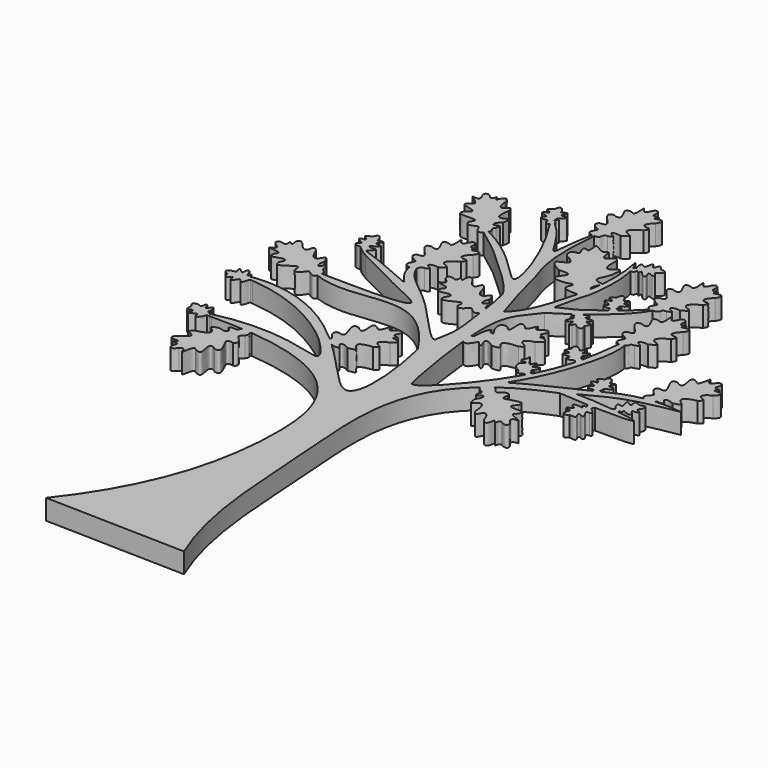
from build123d import *

# Parameters (mm, degrees)
F1_DEPTH = 2


with BuildPart() as f1:
    # F0 (on Top) → F1 (new body)
    with BuildSketch(Plane.XY):
        with BuildLine():
            add(Edge.make_bspline(
                [(-7.2830244899, 23.8568969071), (-6.9255950182, 23.6186106338), (-6.6003847978, 23.3645522922), (-6.3044011406, 23.1031627044)],
                knots=[0, 0, 0, 0, 0.0682019053, 0.0682019053, 0.0682019053, 0.0682019053], degree=3))
            add(Edge.make_bspline(
                [(-7.2830244899, 23.8568969071), (-6.9994019887, 23.4828891588), (-6.7269258202, 23.0977950442), (-6.4662523853, 22.7063580958)],
                knots=[0, 0, 0, 0, 0.0462747937, 0.0462747937, 0.0462747937, 0.0462747937], degree=3))
            add(Edge.make_bspline(
                [(-6.3044011387, 23.103162705), (-6.3084104619, 22.9629474152), (-6.367535654, 22.7963420103), (-6.4662523853, 22.7063580958)],
                knots=[0.5431885819, 0.5431885819, 0.5431885819, 0.5431885819, 0.7562684626, 0.7562684626, 0.7562684626, 0.7562684626], degree=3))
        make_face()
        with BuildLine():
            add(Edge.make_bspline(
                [(-7.2830244899, 23.8568969071), (-6.9994019887, 23.4828891588), (-6.7269258202, 23.0977950442), (-6.4662523853, 22.7063580958)],
                knots=[0, 0, 0, 0, 0.0462747937, 0.0462747937, 0.0462747937, 0.0462747937], degree=3))
            add(Edge.make_bspline(
                [(-7.2830244899, 23.8568969071), (-6.9255950182, 23.6186106338), (-6.6003847978, 23.3645522922), (-6.3044011406, 23.1031627044)],
                knots=[0, 0, 0, 0, 0.0682019053, 0.0682019053, 0.0682019053, 0.0682019053], degree=3))
            add(Edge.make_bspline(
                [(-6.3550009233, 23.6979370432), (-6.8497508486, 23.2818596451), (-6.3691734412, 23.5006786563), (-6.3021983143, 23.1802005578), (-6.3044011387, 23.103162705)],
                knots=[0, 0, 0, 0, 0.4261170663, 0.5431885819, 0.5431885819, 0.5431885819, 0.5431885819], degree=3))
            add(Edge.make_bspline(
                [(-6.3317185735, 24.4604900705), (-5.9522282507, 24.4901670918), (-6.2356144219, 23.980329772), (-6.9052247039, 23.7305665354), (-6.3550009233, 23.6979370432)],
                knots=[0, 0, 0, 0, 0.544899328, 1, 1, 1, 1], degree=3))
            add(Edge.make_bspline(
                [(-6.7744867176, 24.9365105731), (-6.2490038479, 25.195007756), (-7.04025385, 24.1893972098), (-6.4820505689, 24.4384026276), (-6.3317185735, 24.4604900705)],
                knots=[0, 0, 0, 0, 0.523731518, 1, 1, 1, 1], degree=3))
            add(Edge.make_bspline(
                [(-7.7400428373, 24.9370211106), (-7.707410386, 25.6862208089), (-6.9617080418, 25.0381631981), (-7.0797636203, 24.6748653086), (-6.7744867176, 24.9365105731)],
                knots=[0, 0, 0, 0, 0.5549507788, 1, 1, 1, 1], degree=3))
            add(Edge.make_bspline(
                [(-7.7400428373, 24.9370211106), (-8.4433206567, 24.4842038124), (-7.9152038186, 24.4505832605), (-7.5912267279, 24.1744325854), (-7.9850055517, 24.0789462742)],
                knots=[0, 0, 0, 0, 0.5862987098, 1, 1, 1, 1], degree=3))
            add(Edge.make_bspline(
                [(-7.9850055517, 24.0789462742), (-8.428364221, 23.8879029616), (-7.5828387245, 23.6796045843), (-7.410690254, 23.5855856282), (-7.6697452574, 23.3444934771)],
                knots=[0, 0, 0, 0, 0.5327955397, 1, 1, 1, 1], degree=3))
            add(Edge.make_bspline(
                [(-7.6697452574, 23.3444934771), (-7.8546850708, 23.1254471141), (-7.1553204538, 23.0155870065), (-6.9632573871, 23.2023815112), (-6.9371741265, 22.8524948747)],
                knots=[0, 0, 0, 0, 0.520908595, 1, 1, 1, 1], degree=3))
            add(Edge.make_bspline(
                [(-6.4662523853, 22.7063580958), (-6.5791695722, 22.6034299462), (-6.7438880941, 22.6007529001), (-6.9371741265, 22.8524948747)],
                knots=[0.7562684626, 0.7562684626, 0.7562684626, 0.7562684626, 1, 1, 1, 1], degree=3))
        make_face()
        with BuildLine():
            add(Edge.make_bspline(
                [(-6.3044011387, 23.103162705), (-6.3084104619, 22.9629474152), (-6.367535654, 22.7963420103), (-6.4662523853, 22.7063580958)],
                knots=[0.5431885819, 0.5431885819, 0.5431885819, 0.5431885819, 0.7562684626, 0.7562684626, 0.7562684626, 0.7562684626], degree=3))
            add(Edge.make_bspline(
                [(-6.4662523853, 22.7063580958), (-3.8338543067, 18.7534509981), (-1.0796397982, 9.8866138409), (-5.309965066, 16.7686890167), (-9.3709632135, 18.7661565859)],
                knots=[0.0462747937, 0.0462747937, 0.0462747937, 0.0462747937, 0.51357856, 0.9470877335, 0.9470877335, 0.9470877335, 0.9470877335], degree=3))
            add(Edge.make_bspline(
                [(-9.6069315552, 18.4363055281), (-9.5084751471, 18.5324280861), (-9.4240206604, 18.6535214214), (-9.3709632369, 18.7661565965)],
                knots=[0.321879146, 0.321879146, 0.321879146, 0.321879146, 0.4682971672, 0.4682971672, 0.4682971672, 0.4682971672], degree=3))
            add(Edge.make_bspline(
                [(-9.6069315552, 18.4363055281), (-6.7127627923, 16.2861504157), (-7.5033975813, 16.7226051452), (-2.4754665792, 12.4432705343), (-1.9912521821, 11.2327341922)],
                knots=[0.0587910513, 0.0587910513, 0.0587910513, 0.0587910513, 0.4997982199, 1, 1, 1, 1], degree=3))
            add(Edge.make_bspline(
                [(-1.9912521821, 11.2327341922), (-1.7478000221, 10.3645500172), (-1.6029765018, 9.4526665618), (-1.493116535, 8.5900831123)],
                knots=[0, 0, 0, 0, 0.2731869597, 0.2731869597, 0.2731869597, 0.2731869597], degree=3))
            add(Edge.make_bspline(
                [(-1.4055366788, 7.8606911441), (-1.3348395827, 8.0601358248), (-1.3086866339, 8.4371577768), (-1.4399830487, 8.5541442196), (-1.493116535, 8.5900831123)],
                knots=[0.3298039714, 0.3298039714, 0.3298039714, 0.3298039714, 0.5534606992, 0.6905710429, 0.6905710429, 0.6905710429, 0.6905710429], degree=3))
            add(Edge.make_bspline(
                [(-1.4055366697, 7.860691143), (-1.3932214045, 7.7535636466), (-1.3811860549, 7.6477133218), (-1.3692920143, 7.5433426392)],
                knots=[0.3517115317, 0.3517115317, 0.3517115317, 0.3517115317, 0.3871183948, 0.3871183948, 0.3871183948, 0.3871183948], degree=3))
            add(Edge.make_bspline(
                [(-1.3692920143, 7.5433426392), (-1.3252733715, 7.1570772842), (-1.1284437453, 5.4452417025), (-0.8202554891, 4.4012602884), (-1.2849295745, 2.2735432722)],
                knots=[0.3871183948, 0.3871183948, 0.3871183948, 0.3871183948, 0.5181556188, 1, 1, 1, 1], degree=3))
            add(Edge.make_bspline(
                [(-9.8891811582, 10.4983452218), (-9.3357717416, 8.9759053827), (-5.8907166996, 7.2895616824), (-1.2849295745, 1.1507440358), (-1.2849295745, 2.2735432722)],
                knots=[0.1095027317, 0.1095027317, 0.1095027317, 0.1095027317, 0.5062510293, 1, 1, 1, 1], degree=3))
            add(Edge.make_bspline(
                [(-10.4510760299, 10.3369036325), (-10.2571338112, 10.3316612875), (-10.0108240326, 10.3853016056), (-9.905364039, 10.4796413932), (-9.8891811582, 10.4983452218)],
                knots=[0.3496575833, 0.3496575833, 0.3496575833, 0.3496575833, 0.5533057721, 0.6004182071, 0.6004182071, 0.6004182071, 0.6004182071], degree=3))
            add(Edge.make_bspline(
                [(-10.4510760294, 10.3369036355), (-10.3140219455, 9.1099021242), (-7.6653586081, 7.0333389758), (-11.6802298368, 9.2922770134), (-14.7025460105, 10.2836822372)],
                knots=[0.1183888662, 0.1183888662, 0.1183888662, 0.1183888662, 0.4210143149, 0.9201006341, 0.9201006341, 0.9201006341, 0.9201006341], degree=3))
            add(Edge.make_bspline(
                [(-14.7025460105, 10.2836822372), (-14.7673833856, 10.3049507309), (-14.8324614381, 10.3260283034), (-14.897759835, 10.3468942704)],
                knots=[0.9201006341, 0.9201006341, 0.9201006341, 0.9201006341, 0.9308074712, 0.9308074712, 0.9308074712, 0.9308074712], degree=3))
            add(Edge.make_bspline(
                [(-14.897759835, 10.3468942704), (-14.9727316961, 10.2937614568), (-15.0386428159, 10.2505367323), (-15.0968016872, 10.2175015052)],
                knots=[0.5018258113, 0.5018258113, 0.5018258113, 0.5018258113, 0.5980783923, 0.5980783923, 0.5980783923, 0.5980783923], degree=3))
            ThreePointArc((-15.0968016872, 10.2175015052), (-14.7461259396, 9.9703089804), (-14.3755495259, 9.7540897725))
            add(Edge.make_bspline(
                [(-14.3755495259, 9.7540897725), (-8.9747821887, 6.9062057993), (-6.3313092697, 6.1282188527), (-6.1021251578, 4.9786287609), (-15.0424187755, 5.192235557)],
                knots=[0.0481512352, 0.0481512352, 0.0481512352, 0.0481512352, 0.5137757923, 0.9808881786, 0.9808881786, 0.9808881786, 0.9808881786], degree=3))
            add(Edge.make_bspline(
                [(-15.1383101255, 4.7517992821), (-15.0745436105, 4.8761570065), (-15.0440617061, 5.040322544), (-15.0424187735, 5.192235557)],
                knots=[0.250044121, 0.250044121, 0.250044121, 0.250044121, 0.4133131161, 0.4133131161, 0.4133131161, 0.4133131161], degree=3))
            add(Edge.make_bspline(
                [(-15.1383101255, 4.7517992821), (-12.7532848253, 3.8774020861), (-8.0868188911, 5.1006038753), (-4.2323740655, 4.3790526224), (-1.3530709548, -0.0416957773)],
                knots=[0.0604344916, 0.0604344916, 0.0604344916, 0.0604344916, 0.4807848396, 1, 1, 1, 1], degree=3))
            add(Edge.make_bspline(
                [(-1.3530709548, -0.0416957773), (-0.4063348806, -3.934545887), (0.2828604309, -12.498539455), (-4.3181311542, -6.1754022999), (-7.0428329479, -3.6007162315)],
                knots=[0, 0, 0, 0, 0.3884589782, 0.6606793216, 0.6606793216, 0.6606793216, 0.6606793216], degree=3))
            add(Edge.make_bspline(
                [(-8.328963206, -3.5805012004), (-8.1353376019, -3.6183404142), (-7.5871997753, -3.5075285988), (-7.0428329479, -3.6007162315)],
                knots=[0.5465429425, 0.5465429425, 0.5465429425, 0.5465429425, 1.2981362677, 1.2981362677, 1.2981362677, 1.2981362677], degree=3))
            add(Edge.make_bspline(
                [(-8.328963206, -3.5805012004), (-7.2743808376, -4.5386566954), (-5.0966495142, -7.5286586899), (-10.6621504134, -3.916051762), (-17.2697339143, -5.3783508986)],
                knots=[0.3673838243, 0.3673838243, 0.3673838243, 0.3673838243, 0.530952326, 0.9642641358, 0.9642641358, 0.9642641358, 0.9642641358], degree=3))
            add(Edge.make_bspline(
                [(-17.2697339143, -5.3783508986), (-17.0699147841, -5.4490751014), (-16.8737823844, -5.7399924552), (-17.2020280737, -5.7858311085)],
                knots=[0.5510318037, 0.5510318037, 0.5510318037, 0.5510318037, 0.9395322665, 0.9395322665, 0.9395322665, 0.9395322665], degree=3))
            add(Edge.make_bspline(
                [(-17.2020280737, -5.7858311085), (-16.0389379646, -5.7769651924), (-14.9585359339, -5.8085371052), (-13.9550962522, -5.8773551655)],
                knots=[0.0188984067, 0.0188984067, 0.0188984067, 0.0188984067, 0.0578050771, 0.0578050771, 0.0578050771, 0.0578050771], degree=3))
            add(Edge.make_bspline(
                [(-13.5841550604, -5.9047626628), (-13.7152164046, -5.8729392418), (-13.8501737569, -5.8633114215), (-13.9550962522, -5.8773551655)],
                knots=[0.3706410184, 0.3706410184, 0.3706410184, 0.3706410184, 0.5120718061, 0.5120718061, 0.5120718061, 0.5120718061], degree=3))
            add(Edge.make_bspline(
                [(-13.5841550604, -5.9047626628), (-13.4170183881, -5.9180123118), (-13.2520798732, -5.9323242566), (-13.0893114899, -5.9476828747)],
                knots=[0.0626453243, 0.0626453243, 0.0626453243, 0.0626453243, 0.0692512465, 0.0692512465, 0.0692512465, 0.0692512465], degree=3))
            add(Edge.make_bspline(
                [(-13.0893114899, -5.9476828747), (-2.2991147312, -6.9658321487), (0.3647541555, -18.9059884875), (-3.1700518728, -31.0652612365), (-8.2570081856, -37.4728685832)],
                knots=[0.0692512465, 0.0692512465, 0.0692512465, 0.0692512465, 0.507169219, 1, 1, 1, 1], degree=3))
            Line((-8.2570081856, -37.4728685832), (5.6844632793, -37.8173051989))
            add(Edge.make_bspline(
                [(6.446316549, -1.9733819286), (1.2529114407, -6.3985529422), (3.1303302028, -20.1557258024), (2.9898207168, -31.3916216107), (5.6844632793, -37.8173051989)],
                knots=[0.1055909767, 0.1055909767, 0.1055909767, 0.1055909767, 0.5110738844, 1, 1, 1, 1], degree=3))
            add(Edge.make_bspline(
                [(7.2087163952, -1.3694859015), (6.831004006, -1.3391741179), (6.4930997677, -1.6920472218), (6.446316549, -1.9733819286)],
                knots=[0.1037976926, 0.1037976926, 0.1037976926, 0.1037976926, 0.4679233051, 0.4679233051, 0.4679233051, 0.4679233051], degree=3))
            add(Edge.make_bspline(
                [(11.8472744276, 1.073961144), (9.9682824961, 0.3626392861), (8.4432034603, -0.4594564005), (7.2087163963, -1.3694859064)],
                knots=[0, 0, 0, 0, 0.086781452, 0.086781452, 0.086781452, 0.086781452], degree=3))
            add(Edge.make_bspline(
                [(11.8472744276, 1.073961144), (12.8342047056, 0.988598542), (13.8322293089, 0.9274083452), (14.761860181, 0.888550806)],
                knots=[0, 0, 0, 0, 0.1325939353, 0.1325939353, 0.1325939353, 0.1325939353], degree=3))
            add(Edge.make_bspline(
                [(14.7618601827, 0.8885508054), (14.8122427021, 1.1702791042), (15.5318953014, 1.5872043624), (15.4721919876, 0.8627236551)],
                knots=[0.4417596054, 0.4417596054, 0.4417596054, 0.4417596054, 1, 1, 1, 1], degree=3))
            add(Edge.make_bspline(
                [(15.4721919876, 0.8627236551), (17.8372520288, 0.7899058738), (20.4429230326, 0.9130749251), (18.241283581, 1.3074177908), (17.3314129646, 1.4290121267)],
                knots=[0.1670925821, 0.1670925821, 0.1670925821, 0.1670925821, 0.5199750669, 0.6973219139, 0.6973219139, 0.6973219139, 0.6973219139], degree=3))
            add(Edge.make_bspline(
                [(17.3314129646, 1.4290121267), (17.3437413917, 1.3859183147), (17.3914206373, 1.070297292), (16.3993047386, 0.8138388359), (16.6502745462, 1.5143461557)],
                knots=[0.3273741769, 0.3273741769, 0.3273741769, 0.3273741769, 0.428573246, 1, 1, 1, 1], degree=3))
            add(Edge.make_bspline(
                [(16.6502745462, 1.5143461557), (15.2246778839, 1.6819377737), (13.6143610425, 1.8063747813), (12.9679338421, 1.7595318073)],
                knots=[0.7399514284, 0.7399514284, 0.7399514284, 0.7399514284, 1, 1, 1, 1], degree=3))
            add(Edge.make_bspline(
                [(12.9679338421, 1.7595318073), (14.0693364398, 2.3616779206), (16.4055643867, 3.6388875634), (19.5145668442, 4.1801976876), (21.1578458548, 4.4663053704)],
                knots=[0, 0, 0, 0, 0.4714455657, 1, 1, 1, 1], degree=3))
            add(Edge.make_bspline(
                [(18.4401991516, 4.5747355467), (19.2408398991, 4.6411299893), (20.1338213578, 4.6171305666), (21.1578458548, 4.4663053704)],
                knots=[0.8559667545, 0.8559667545, 0.8559667545, 0.8559667545, 1, 1, 1, 1], degree=3))
            add(Edge.make_bspline(
                [(17.4734380729, 4.4452043984), (17.6901900529, 4.3148910325), (18.3083682643, 4.2362771463), (18.3714417845, 4.492748455), (18.4401991516, 4.5747355467)],
                knots=[0.2654447151, 0.2654447151, 0.2654447151, 0.2654447151, 0.5533057721, 0.792791285, 0.792791285, 0.792791285, 0.792791285], degree=3))
            add(Edge.make_bspline(
                [(14.1640380219, 3.2511269768), (15.1731715133, 3.748057022), (16.2091915948, 4.2092589897), (17.4734380729, 4.4452043984)],
                knots=[0.5456420171, 0.5456420171, 0.5456420171, 0.5456420171, 0.7952127199, 0.7952127199, 0.7952127199, 0.7952127199], degree=3))
            add(Edge.make_bspline(
                [(14.1640380219, 3.2511269768), (14.1860857829, 3.2361228299), (14.3855197396, 3.0467106298), (13.8975782977, 2.2887752246), (13.5501283214, 2.9451712436)],
                knots=[0.368500824, 0.368500824, 0.368500824, 0.368500824, 0.4296677883, 1, 1, 1, 1], degree=3))
            add(Edge.make_bspline(
                [(7.5175091624, -0.09986246), (9.3350757417, 0.9817453369), (11.4605001227, 1.9013735083), (13.4589560476, 2.899552344), (13.5501283214, 2.9451712436)],
                knots=[0, 0, 0, 0, 0.4722911355, 0.4948975859, 0.4948975859, 0.4948975859, 0.4948975859], degree=3))
            add(Edge.make_bspline(
                [(10.7582724372, 10.4403925304), (11.0580887415, 8.8951649854), (9.7997969923, 3.9653101335), (8.4524664697, 1.4318507999), (7.5175091624, -0.09986246)],
                knots=[0.0980497672, 0.0980497672, 0.0980497672, 0.0980497672, 0.5259226462, 1, 1, 1, 1], degree=3))
            add(Edge.make_bspline(
                [(10.2860692098, 10.3784734911), (10.453312226, 10.3652586853), (10.6325102245, 10.3907018842), (10.7582724372, 10.4403925304)],
                knots=[0.3298039803, 0.3298039803, 0.3298039803, 0.3298039803, 0.5071239237, 0.5071239237, 0.5071239237, 0.5071239237], degree=3))
            add(Edge.make_bspline(
                [(10.2860692099, 10.3784734944), (10.127456281, 9.0214651429), (9.9705823621, 7.7856493446), (9.6945917347, 6.5660976988)],
                knots=[0.0483655939, 0.0483655939, 0.0483655939, 0.0483655939, 0.2531433198, 0.2531433198, 0.2531433198, 0.2531433198], degree=3))
            add(Edge.make_bspline(
                [(9.694591745, 6.5660977083), (9.7247752432, 6.5474523657), (10.044472416, 6.3081206624), (10.1297895815, 5.488774521), (9.5148742232, 5.8396972126)],
                knots=[0.4006505727, 0.4006505727, 0.4006505727, 0.4006505727, 0.4563375845, 1, 1, 1, 1], degree=3))
            add(Edge.make_bspline(
                [(9.5148742232, 5.8396972126), (9.2084454063, 4.7030046056), (8.7771848182, 3.5623003099), (8.122674161, 2.3321363656)],
                knots=[0.2938623185, 0.2938623185, 0.2938623185, 0.2938623185, 0.4850906625, 0.4850906625, 0.4850906625, 0.4850906625], degree=3))
            add(Edge.make_bspline(
                [(8.1226741606, 2.3321363672), (8.1488482126, 2.3298892749), (8.4376135787, 2.2578745974), (8.5439890995, 1.2950675968), (7.8989630376, 1.6631482565)],
                knots=[0.372790437, 0.372790437, 0.372790437, 0.372790437, 0.4296860012, 1, 1, 1, 1], degree=3))
            add(Edge.make_bspline(
                [(7.8228000039, 1.7897509333), (7.8465768524, 1.7582273046), (7.8716474696, 1.7167151278), (7.8989630376, 1.6631482565)],
                knots=[0.9177938546, 0.9177938546, 0.9177938546, 0.9177938546, 1, 1, 1, 1], degree=3))
            add(Edge.make_bspline(
                [(7.8228000039, 1.7897509333), (7.816996451, 1.7796320131), (5.9742818835, -1.4268766538), (2.5850140554, -5.2989103696), (1.9143626357, -4.861554145)],
                knots=[0.5128877349, 0.5128877349, 0.5128877349, 0.5128877349, 0.5144259379, 1, 1, 1, 1], degree=3))
            add(Edge.make_bspline(
                [(0.5761754001, 3.1602606177), (0.9451592299, -0.7970737273), (1.9143626357, -5.449141318), (1.9143626357, -4.861554145)],
                knots=[0.5407383011, 0.5407383011, 0.5407383011, 0.5407383011, 1, 1, 1, 1], degree=3))
            add(Edge.make_bspline(
                [(0.356165784, 4.1867696999), (0.1430285645, 3.7735971671), (0.3180393897, 3.3434200247), (0.5761754001, 3.1602606177)],
                knots=[0, 0, 0, 0, 0.3538981495, 0.3538981495, 0.3538981495, 0.3538981495], degree=3))
            add(Edge.make_bspline(
                [(0.4879269392, 4.2749555028), (0.4505111657, 4.2494053471), (0.406920597, 4.2203901767), (0.3561657844, 4.1867697008)],
                knots=[0.9504400513, 0.9504400513, 0.9504400513, 0.9504400513, 1, 1, 1, 1], degree=3))
            add(Edge.make_bspline(
                [(2.5086239283, 10.8435213137), (1.6155901987, 9.542235904), (0.365514994, 8.923768042), (0.4308962718, 5.1730894013), (0.4879269479, 4.2749554964)],
                knots=[0, 0, 0, 0, 0.3872431223, 0.4966718837, 0.4966718837, 0.4966718837, 0.4966718837], degree=3))
            add(Edge.make_bspline(
                [(4.2733086601, 11.9916081706), (3.7609880573, 11.6345058014), (3.1880432336, 11.2608790005), (2.5086239283, 10.8435213137)],
                knots=[0.799561152, 0.799561152, 0.799561152, 0.799561152, 1, 1, 1, 1], degree=3))
            add(Edge.make_bspline(
                [(4.2733086601, 11.9916081706), (4.0926025657, 12.2220839643), (4.0915020215, 12.8892690841), (4.6868465814, 12.5795747609)],
                knots=[0.4846553649, 0.4846553649, 0.4846553649, 0.4846553649, 1, 1, 1, 1], degree=3))
            add(Edge.make_bspline(
                [(4.8352131211, 12.394222602), (4.7939813835, 12.414451534), (4.7485691527, 12.4694215496), (4.6868465814, 12.5795747609)],
                knots=[0.8275837687, 0.8275837687, 0.8275837687, 0.8275837687, 1, 1, 1, 1], degree=3))
            add(Edge.make_bspline(
                [(8.8046101757, 16.3757008495), (8.151493883, 15.206340136), (6.7168744867, 13.8735208208), (5.3718904324, 12.7897850181), (4.8352131211, 12.394222602)],
                knots=[0.0870296928, 0.0870296928, 0.0870296928, 0.0870296928, 0.4956337185, 0.7231675212, 0.7231675212, 0.7231675212, 0.7231675212], degree=3))
            add(Edge.make_bspline(
                [(8.5336353676, 16.3924189922), (8.6194799745, 16.3752356234), (8.7132966298, 16.3704375949), (8.8046101773, 16.3757008456)],
                knots=[0.2888816238, 0.2888816238, 0.2888816238, 0.2888816238, 0.3852069167, 0.3852069167, 0.3852069167, 0.3852069167], degree=3))
            add(Edge.make_bspline(
                [(6.6940593459, 14.7283197348), (7.2847427727, 15.193027485), (7.9313144002, 15.7391139113), (8.5336353689, 16.3924189828)],
                knots=[0.6374849498, 0.6374849498, 0.6374849498, 0.6374849498, 0.9016899501, 0.9016899501, 0.9016899501, 0.9016899501], degree=3))
            add(Edge.make_bspline(
                [(6.6940593459, 14.7283197348), (6.8129180716, 14.4820206348), (6.5371498988, 13.7807316739), (6.1166912345, 14.2829045348)],
                knots=[0.4501673847, 0.4501673847, 0.4501673847, 0.4501673847, 0.9882075126, 0.9882075126, 0.9882075126, 0.9882075126], degree=3))
            add(Edge.make_bspline(
                [(2.5045169245, 12.0716887873), (4.3400707655, 12.8143043257), (4.8825294689, 13.3450848026), (5.9466513405, 14.1533197636), (6.1166912345, 14.2829045348)],
                knots=[0, 0, 0, 0, 0.4649552007, 0.5479499639, 0.5479499639, 0.5479499639, 0.5479499639], degree=3))
            add(Edge.make_bspline(
                [(3.3222327634, 20.4571259636), (3.7925422208, 18.6439709734), (3.2355094619, 14.0648635936), (3.2344385937, 15.5560774729), (2.5045169245, 12.0716887873)],
                knots=[0.1235301969, 0.1235301969, 0.1235301969, 0.1235301969, 0.5693789902, 1, 1, 1, 1], degree=3))
            add(Edge.make_bspline(
                [(3.3222327601, 20.4571259541), (3.0594839142, 20.4745750447), (2.7856077676, 20.6611324054), (3.1430146194, 21.0221629646)],
                knots=[0.6098746192, 0.6098746192, 0.6098746192, 0.6098746192, 1, 1, 1, 1], degree=3))
            add(Edge.make_bspline(
                [(2.7386521356, 21.8009612559), (2.900752588, 21.5693892879), (3.0340854306, 21.3064074696), (3.1430146194, 21.0221629646)],
                knots=[0, 0, 0, 0, 0.0755321584, 0.0755321584, 0.0755321584, 0.0755321584], degree=3))
            add(Edge.make_bspline(
                [(2.7386521356, 21.8009612559), (3.0752467313, 20.1581892326), (3.1121986134, 18.7410877316), (2.9803331122, 17.4184252629)],
                knots=[0, 0, 0, 0, 0.2884123735, 0.2884123735, 0.2884123735, 0.2884123735], degree=3))
            add(Edge.make_bspline(
                [(3.0635552921, 17.4066587767), (3.0350801461, 17.4105759006), (3.0073431659, 17.4144942674), (2.9803331107, 17.4184252552)],
                knots=[0, 0, 0, 0, 0.0198410334, 0.0198410334, 0.0198410334, 0.0198410334], degree=3))
            add(Edge.make_bspline(
                [(2.9593425888, 17.2210636735), (2.9908538076, 17.2790319374), (3.0255184086, 17.3407769618), (3.0635552921, 17.4066587767)],
                knots=[0.9657365348, 0.9657365348, 0.9657365348, 0.9657365348, 1, 1, 1, 1], degree=3))
            add(Edge.make_bspline(
                [(2.9593425888, 17.2210636735), (2.9184844432, 16.8593876837), (2.8653229442, 16.5043747361), (2.8025889497, 16.1532854948)],
                knots=[0.3028076768, 0.3028076768, 0.3028076768, 0.3028076768, 0.3822190977, 0.3822190977, 0.3822190977, 0.3822190977], degree=3))
            add(Edge.make_bspline(
                [(2.7378248051, 14.9060022086), (3.2836535405, 15.0361399771), (3.0670694512, 15.7673816922), (2.8374494935, 16.1001542511), (2.8025889497, 16.1532854948)],
                knots=[0, 0, 0, 0, 0.4645235559, 0.5603510205, 0.5603510205, 0.5603510205, 0.5603510205], degree=3))
            add(Edge.make_bspline(
                [(2.5385402672, 14.8949403039), (2.6023877138, 14.897866903), (2.6687898787, 14.901548307), (2.7378248051, 14.9060022086)],
                knots=[0.9710196428, 0.9710196428, 0.9710196428, 0.9710196428, 1, 1, 1, 1], degree=3))
            add(Edge.make_bspline(
                [(2.5385402661, 14.8949403077), (2.4739214801, 14.6221098604), (1.9032979762, 12.3536021444), (1.1545733203, 10.0184055106), (-0.0909709431, 9.0496486414)],
                knots=[0.478021418, 0.478021418, 0.478021418, 0.478021418, 0.5407103431, 1, 1, 1, 1], degree=3))
            add(Edge.make_bspline(
                [(-2.542555068, 23.3056752253), (-3.0504367313, 18.0610177026), (-1.5919461527, 15.2084122789), (-1.4740818718, 13.2681371194), (-0.0909709431, 9.0496486414)],
                knots=[0.0378820958, 0.0378820958, 0.0378820958, 0.0378820958, 0.5436572492, 1, 1, 1, 1], degree=3))
            add(Edge.make_bspline(
                [(-2.7556512283, 23.3163689706), (-2.6846983844, 23.3059393633), (-2.6120665365, 23.3025597195), (-2.5425550635, 23.3056752005)],
                knots=[0.3331169447, 0.3331169447, 0.3331169447, 0.3331169447, 0.4066102753, 0.4066102753, 0.4066102753, 0.4066102753], degree=3))
            add(Edge.make_bspline(
                [(-6.3044011406, 23.1031627044), (-4.3663923691, 21.3916651209), (-3.0540938772, 17.5107071946), (-3.257264777, 21.1724405488), (-2.7556512282, 23.3163689721)],
                knots=[0.0682019053, 0.0682019053, 0.0682019053, 0.0682019053, 0.5147667326, 0.9237135709, 0.9237135709, 0.9237135709, 0.9237135709], degree=3))
        make_face()
        with BuildLine():
            add(Edge.make_bspline(
                [(-9.6069315552, 18.4363055281), (-9.5084751471, 18.5324280861), (-9.4240206604, 18.6535214214), (-9.3709632369, 18.7661565965)],
                knots=[0.321879146, 0.321879146, 0.321879146, 0.321879146, 0.4682971672, 0.4682971672, 0.4682971672, 0.4682971672], degree=3))
            add(Edge.make_bspline(
                [(-9.3709632135, 18.7661565859), (-9.8666311929, 19.0099588922), (-10.3924695903, 19.23417865), (-10.949219577, 19.4297935814)],
                knots=[0.9470877335, 0.9470877335, 0.9470877335, 0.9470877335, 1, 1, 1, 1], degree=3))
            add(Edge.make_bspline(
                [(-10.949219577, 19.4297935814), (-10.4365980989, 19.0514301251), (-9.9927557238, 18.7229445864), (-9.6069315552, 18.4363055281)],
                knots=[0, 0, 0, 0, 0.0587910513, 0.0587910513, 0.0587910513, 0.0587910513], degree=3))
        make_face()
        with BuildLine():
            add(Edge.make_bspline(
                [(-9.3709632135, 18.7661565859), (-9.8666311929, 19.0099588922), (-10.3924695903, 19.23417865), (-10.949219577, 19.4297935814)],
                knots=[0.9470877335, 0.9470877335, 0.9470877335, 0.9470877335, 1, 1, 1, 1], degree=3))
            add(Edge.make_bspline(
                [(-9.3709632369, 18.7661565965), (-9.3401587121, 18.831551273), (-9.2136818404, 19.2227422135), (-9.6344226864, 19.2464536881), (-9.3408973898, 19.6321291082)],
                knots=[0.4682971672, 0.4682971672, 0.4682971672, 0.4682971672, 0.5533057724, 1, 1, 1, 1], degree=3))
            add(Edge.make_bspline(
                [(-9.3408973898, 19.6321291082), (-9.0581260233, 20.3277672421), (-9.9940824129, 19.5406629407), (-9.9851762229, 20.2630250739), (-9.4643028276, 20.6685900495)],
                knots=[0, 0, 0, 0, 0.4354555568, 1, 1, 1, 1], degree=3))
            add(Edge.make_bspline(
                [(-9.4643028276, 20.6685900495), (-9.2801870352, 21.5825599843), (-9.7234967616, 21.2054915308), (-10.6471140566, 20.9087385495), (-10.3259685534, 22.4749946638)],
                knots=[0, 0, 0, 0, 0.4149720401, 1, 1, 1, 1], degree=3))
            add(Edge.make_bspline(
                [(-10.3259685534, 22.4749946638), (-10.4887563334, 23.2134681913), (-10.9544392317, 22.2470909426), (-11.432457287, 22.5909130074), (-11.4738575261, 23.4381878774)],
                knots=[0, 0, 0, 0, 0.4338460012, 1, 1, 1, 1], degree=3))
            add(Edge.make_bspline(
                [(-11.4738575261, 23.4381878774), (-11.7289587585, 24.382018242), (-12.3026097677, 23.3884833436), (-12.2694089579, 23.2256159054), (-12.4794597403, 23.7102036864)],
                knots=[0, 0, 0, 0, 0.5881854472, 1, 1, 1, 1], degree=3))
            add(Edge.make_bspline(
                [(-12.4794597403, 23.7102036864), (-12.7650766323, 22.9625001686), (-13.0461325682, 23.9037740501), (-13.8126212844, 23.6167702057), (-13.4471147419, 22.9873728909)],
                knots=[0, 0, 0, 0, 0.5057015893, 1, 1, 1, 1], degree=3))
            add(Edge.make_bspline(
                [(-13.4471147419, 22.9873728909), (-13.1669183839, 22.3409593834), (-15.0860747741, 23.0669526094), (-12.6786651087, 21.79766709), (-13.3955704458, 21.6500834193)],
                knots=[0, 0, 0, 0, 0.4392164651, 1, 1, 1, 1], degree=3))
            add(Edge.make_bspline(
                [(-13.3955704458, 21.6500834193), (-14.1472438379, 21.0770556006), (-12.7283150396, 21.0124035252), (-12.2892945168, 20.601432118), (-12.9457640514, 20.2494577208)],
                knots=[0, 0, 0, 0, 0.5374091068, 1, 1, 1, 1], degree=3))
            add(Edge.make_bspline(
                [(-12.9457640514, 20.2494577208), (-13.4142689709, 19.619387011), (-11.9253137432, 19.744975993), (-11.1647484884, 19.718013749), (-11.6036168571, 19.123262505)],
                knots=[0, 0, 0, 0, 0.5566164277, 1, 1, 1, 1], degree=3))
            add(Edge.make_bspline(
                [(-11.6036168571, 19.123262505), (-11.640961618, 18.5322561787), (-10.5515227365, 18.9409723743), (-10.4687919136, 19.0386722265), (-10.2744542022, 18.519559423)],
                knots=[0, 0, 0, 0, 0.5487699329, 1, 1, 1, 1], degree=3))
            add(Edge.make_bspline(
                [(-10.2744542022, 18.519559423), (-10.1074844502, 18.1343602059), (-9.8233739321, 18.2249937877), (-9.6069315552, 18.4363055281)],
                knots=[0, 0, 0, 0, 0.321879146, 0.321879146, 0.321879146, 0.321879146], degree=3))
            add(Edge.make_bspline(
                [(-10.949219577, 19.4297935814), (-10.4365980989, 19.0514301251), (-9.9927557238, 18.7229445864), (-9.6069315552, 18.4363055281)],
                knots=[0, 0, 0, 0, 0.0587910513, 0.0587910513, 0.0587910513, 0.0587910513], degree=3))
        make_face()
        with BuildLine():
            add(Edge.make_bspline(
                [(-3.1700518728, 23.9443720662), (-3.3643605659, 23.5557543995), (-3.0772531258, 23.3636423613), (-2.7556512283, 23.3163689706)],
                knots=[0, 0, 0, 0, 0.3331169447, 0.3331169447, 0.3331169447, 0.3331169447], degree=3))
            add(Edge.make_bspline(
                [(-2.7556512282, 23.3163689721), (-2.6620784141, 23.7163051703), (-2.547670603, 24.1299369341), (-2.4062932935, 24.5486311615)],
                knots=[0.9237135709, 0.9237135709, 0.9237135709, 0.9237135709, 1, 1, 1, 1], degree=3))
            add(Edge.make_bspline(
                [(-2.4062932935, 24.5486311615), (-2.4593250113, 24.1123246996), (-2.5045151966, 23.6984952703), (-2.542555068, 23.3056752253)],
                knots=[0, 0, 0, 0, 0.0378820958, 0.0378820958, 0.0378820958, 0.0378820958], degree=3))
            add(Edge.make_bspline(
                [(-2.5425550635, 23.3056752005), (-2.4052999253, 23.3118269301), (-1.8938074348, 23.4405319031), (-2.2035243415, 23.9212366711), (-1.7176952958, 23.9443720662)],
                knots=[0.4066102753, 0.4066102753, 0.4066102753, 0.4066102753, 0.5517278626, 1, 1, 1, 1], degree=3))
            add(Edge.make_bspline(
                [(-1.7176952958, 23.9443720662), (-1.0005143696, 24.1757200964), (-2.2152152441, 24.417521636), (-1.6261425866, 24.7555976322), (-0.982412952, 24.6176552027)],
                knots=[0, 0, 0, 0, 0.4369967049, 1, 1, 1, 1], degree=3))
            add(Edge.make_bspline(
                [(-0.982412952, 24.6176552027), (-0.1639240122, 25.0641028728), (-0.737729205, 25.1613228954), (-1.5587449307, 25.6781056523), (-0.1524947875, 26.438863948)],
                knots=[0, 0, 0, 0, 0.4149720401, 1, 1, 1, 1], degree=3))
            add(Edge.make_bspline(
                [(-0.1524947875, 26.438863948), (0.3085707867, 27.0382482558), (-0.7310523317, 26.7738067306), (-0.7749334327, 27.3609943688), (-0.1524947875, 27.9373265803)],
                knots=[0, 0, 0, 0, 0.4338460012, 1, 1, 1, 1], degree=3))
            add(Edge.make_bspline(
                [(-0.1524947875, 27.9373265803), (0.4065453071, 28.7394279258), (-0.7232823418, 28.5402381712), (-0.8267049686, 28.410115704), (-0.5905072321, 28.8825109601)],
                knots=[0, 0, 0, 0, 0.5881854472, 1, 1, 1, 1], degree=3))
            add(Edge.make_bspline(
                [(-0.5905072321, 28.8825109601), (-1.3468723563, 28.6206916361), (-0.8064740031, 29.4410321624), (-1.519021153, 29.843714069), (-1.7662243918, 29.1591510177)],
                knots=[0, 0, 0, 0, 0.5057015893, 1, 1, 1, 1], degree=3))
            add(Edge.make_bspline(
                [(-1.7662243918, 29.1591510177), (-2.08129912, 28.5290015613), (-2.7587659921, 30.4658200999), (-2.1836420066, 27.8057562984), (-2.7575155254, 28.2600726932)],
                knots=[0, 0, 0, 0, 0.4392164651, 1, 1, 1, 1], degree=3))
            add(Edge.make_bspline(
                [(-2.7575155254, 28.2600726932), (-3.6796466447, 28.4675527364), (-2.8171031573, 27.3390326623), (-2.8497285675, 26.7385561019), (-3.5413270816, 27.0151961595)],
                knots=[0, 0, 0, 0, 0.5374091068, 1, 1, 1, 1], degree=3))
            add(Edge.make_bspline(
                [(-3.5413270816, 27.0151961595), (-4.325138405, 26.9690901041), (-3.2718496915, 25.9092112675), (-2.8036220465, 25.309253484), (-3.5413270816, 25.2631474286)],
                knots=[0, 0, 0, 0, 0.5566164277, 1, 1, 1, 1], degree=3))
            add(Edge.make_bspline(
                [(-3.5413270816, 25.2631474286), (-4.0350410024, 24.8993578923), (-3.0182159768, 24.3210739496), (-2.9091149454, 24.4060303619), (-3.1700518728, 23.9443720662)],
                knots=[0, 0, 0, 0, 0.5683061987, 1, 1, 1, 1], degree=3))
        make_face()
        with BuildLine():
            add(Edge.make_bspline(
                [(-2.7556512282, 23.3163689721), (-2.6620784141, 23.7163051703), (-2.547670603, 24.1299369341), (-2.4062932935, 24.5486311615)],
                knots=[0.9237135709, 0.9237135709, 0.9237135709, 0.9237135709, 1, 1, 1, 1], degree=3))
            add(Edge.make_bspline(
                [(-2.7556512283, 23.3163689706), (-2.6846983844, 23.3059393633), (-2.6120665365, 23.3025597195), (-2.5425550635, 23.3056752005)],
                knots=[0.3331169447, 0.3331169447, 0.3331169447, 0.3331169447, 0.4066102753, 0.4066102753, 0.4066102753, 0.4066102753], degree=3))
            add(Edge.make_bspline(
                [(-2.4062932935, 24.5486311615), (-2.4593250113, 24.1123246996), (-2.5045151966, 23.6984952703), (-2.542555068, 23.3056752253)],
                knots=[0, 0, 0, 0, 0.0378820958, 0.0378820958, 0.0378820958, 0.0378820958], degree=3))
        make_face()
        with BuildLine():
            add(Edge.make_bspline(
                [(-1.4055366788, 7.8606911441), (-1.3348395827, 8.0601358248), (-1.3086866339, 8.4371577768), (-1.4399830487, 8.5541442196), (-1.493116535, 8.5900831123)],
                knots=[0.3298039714, 0.3298039714, 0.3298039714, 0.3298039714, 0.5534606992, 0.6905710429, 0.6905710429, 0.6905710429, 0.6905710429], degree=3))
            add(Edge.make_bspline(
                [(-1.493116535, 8.5900831123), (-1.4615385018, 8.3421430338), (-1.4328491976, 8.0982761784), (-1.4055366697, 7.860691143)],
                knots=[0.2731869597, 0.2731869597, 0.2731869597, 0.2731869597, 0.3517115317, 0.3517115317, 0.3517115317, 0.3517115317], degree=3))
        make_face()
        with BuildLine():
            add(Edge.make_bspline(
                [(-1.493116535, 8.5900831123), (-1.4615385018, 8.3421430338), (-1.4328491976, 8.0982761784), (-1.4055366697, 7.860691143)],
                knots=[0.2731869597, 0.2731869597, 0.2731869597, 0.2731869597, 0.3517115317, 0.3517115317, 0.3517115317, 0.3517115317], degree=3))
            add(Edge.make_bspline(
                [(-1.493116535, 8.5900831123), (-1.6130275411, 8.6711895683), (-1.7494095338, 8.7088923414), (-1.6780375353, 9.0369479388)],
                knots=[0.6905710429, 0.6905710429, 0.6905710429, 0.6905710429, 1, 1, 1, 1], degree=3))
            add(Edge.make_bspline(
                [(-1.6780375353, 9.0369479388), (-1.7157394967, 9.7867250927), (-2.2314201686, 8.677765127), (-2.5289518788, 9.3369929973), (-2.2282208446, 9.9248048123)],
                knots=[0, 0, 0, 0, 0.4353455574, 1, 1, 1, 1], degree=3))
            add(Edge.make_bspline(
                [(-2.2282208446, 9.9248048123), (-2.4476156534, 10.8309535774), (-2.6900346962, 10.3018627159), (-3.4017030138, 9.6425756424), (-3.7725747799, 11.1978077095)],
                knots=[0, 0, 0, 0, 0.4149720401, 1, 1, 1, 1], degree=3))
            add(Edge.make_bspline(
                [(-3.7725747799, 11.1978077095), (-4.232203011, 11.7982949295), (-4.245846375, 10.7256536068), (-4.8243833443, 10.8352430618), (-5.2199785361, 11.5856383771)],
                knots=[0, 0, 0, 0, 0.4338460012, 1, 1, 1, 1], degree=3))
            add(Edge.make_bspline(
                [(-5.2199785361, 11.5856383771), (-5.8500587176, 12.3332287468), (-5.9500771025, 11.1903449393), (-5.8511561964, 11.0567681804), (-6.2463225019, 11.4071825632)],
                knots=[0, 0, 0, 0, 0.5881854472, 1, 1, 1, 1], degree=3))
            add(Edge.make_bspline(
                [(-6.2463225019, 11.4071825632), (-6.1891861542, 10.6088261283), (-6.8417088691, 11.3431306058), (-7.4150904954, 10.7590846578), (-6.8178342706, 10.3431267099)],
                knots=[0, 0, 0, 0, 0.5057015893, 1, 1, 1, 1], degree=3))
            add(Edge.make_bspline(
                [(-6.8178342706, 10.3431267099), (-6.2907039765, 9.8756932121), (-8.3368683528, 9.7225959886), (-5.6185909866, 9.5896479264), (-6.2059563218, 9.1529144091)],
                knots=[0, 0, 0, 0, 0.4392164651, 1, 1, 1, 1], degree=3))
            add(Edge.make_bspline(
                [(-6.2059563218, 9.1529144091), (-6.6450317497, 8.3159039324), (-5.3317223828, 8.8569744753), (-4.7601506426, 8.6700459789), (-5.2063632858, 8.0736128283)],
                knots=[0, 0, 0, 0, 0.5374091068, 1, 1, 1, 1], degree=3))
            add(Edge.make_bspline(
                [(-5.2063632858, 8.0736128283), (-5.3646935545, 7.3045761029), (-4.0683180344, 8.0476580454), (-3.3676170847, 8.3446507196), (-3.5140141678, 7.6201492488)],
                knots=[0, 0, 0, 0, 0.5566164277, 1, 1, 1, 1], degree=3))
            add(Edge.make_bspline(
                [(-3.5140141678, 7.6201492488), (-3.2981216645, 7.068814028), (-2.4831997906, 7.901020703), (-2.4499539633, 8.0208820143), (-2.0543669795, 7.6324673329)],
                knots=[0, 0, 0, 0, 0.5486893287, 1, 1, 1, 1], degree=3))
            add(Edge.make_bspline(
                [(-2.0543669795, 7.6324673329), (-1.8416907534, 7.4438703762), (-1.6723003071, 7.4757500481), (-1.5517736179, 7.6039322632)],
                knots=[0, 0, 0, 0, 0.2179260119, 0.2179260119, 0.2179260119, 0.2179260119], degree=3))
            add(Edge.make_bspline(
                [(-1.5517736179, 7.6039322632), (-1.489898122, 7.6697379215), (-1.4409009039, 7.7609245772), (-1.4055366788, 7.8606911441)],
                knots=[0.2179260119, 0.2179260119, 0.2179260119, 0.2179260119, 0.3298039714, 0.3298039714, 0.3298039714, 0.3298039714], degree=3))
        make_face()
        with BuildLine():
            add(Edge.make_bspline(
                [(0.6444998631, 15.8217528672), (1.5351273072, 16.1194883173), (0.8479407313, 15.2582015465), (1.2215068774, 14.8345709553), (2.5385402672, 14.8949403039)],
                knots=[0, 0, 0, 0, 0.3732181626, 0.9710196428, 0.9710196428, 0.9710196428, 0.9710196428], degree=3))
            add(Edge.make_bspline(
                [(2.8025889497, 16.1532854948), (2.7269063569, 15.729729745), (2.6372918338, 15.3118846066), (2.5385402661, 14.8949403077)],
                knots=[0.3822190977, 0.3822190977, 0.3822190977, 0.3822190977, 0.478021418, 0.478021418, 0.478021418, 0.478021418], degree=3))
            add(Edge.make_bspline(
                [(2.8025889497, 16.1532854948), (2.6551159936, 16.3780502491), (2.5865200632, 16.5352166838), (2.9593425888, 17.2210636735)],
                knots=[0.5603510205, 0.5603510205, 0.5603510205, 0.5603510205, 0.9657365348, 0.9657365348, 0.9657365348, 0.9657365348], degree=3))
            add(Edge.make_bspline(
                [(2.9803331122, 17.4184252629), (2.9737514116, 17.3524082363), (2.9667491481, 17.2866264791), (2.9593425888, 17.2210636735)],
                knots=[0.2884123735, 0.2884123735, 0.2884123735, 0.2884123735, 0.3028076768, 0.3028076768, 0.3028076768, 0.3028076768], degree=3))
            add(Edge.make_bspline(
                [(2.9803331107, 17.4184252552), (2.3801680068, 17.5057720476), (1.8437893508, 17.713819049), (2.4718677803, 18.569656303), (2.5895095294, 19.1445023752)],
                knots=[0.0198410334, 0.0198410334, 0.0198410334, 0.0198410334, 0.4607100278, 1, 1, 1, 1], degree=3))
            add(Edge.make_bspline(
                [(2.5895095294, 19.1445023752), (2.8377003677, 20.6117780076), (1.7205723449, 19.2091910592), (1.3313163006, 19.7777469576), (1.4243051938, 21.0684189091)],
                knots=[0, 0, 0, 0, 0.4360827499, 1, 1, 1, 1], degree=3))
            add(Edge.make_bspline(
                [(1.4243051938, 21.0684189091), (1.1830046964, 21.7800846516), (0.6337929728, 20.7028410613), (0.2353351202, 20.8763789962), (0.1318271224, 21.3886961662)],
                knots=[0, 0, 0, 0, 0.5222244908, 1, 1, 1, 1], degree=3))
            add(Edge.make_bspline(
                [(0.1318271224, 21.3886961662), (0.1442160882, 22.2718114023), (-0.2252249466, 20.9254641083), (-1.5915728353, 22.5921643677), (-1.3491865375, 21.7512723735)],
                knots=[0, 0, 0, 0, 0.4296724583, 1, 1, 1, 1], degree=3))
            add(Edge.make_bspline(
                [(-1.3491865375, 21.7512723735), (-1.4482974419, 21.6487672659), (-1.0555627446, 20.7335891019), (-2.0741707027, 21.4948037554), (-1.8011244889, 20.7610128366)],
                knots=[0, 0, 0, 0, 0.5121482306, 1, 1, 1, 1], degree=3))
            add(Edge.make_bspline(
                [(-1.8011244889, 20.7610128366), (-1.3877466492, 20.1629658469), (-2.4574501733, 20.5734909694), (-2.4348232256, 19.4098264667), (-1.7793745006, 19.2310604121)],
                knots=[0, 0, 0, 0, 0.4355610088, 1, 1, 1, 1], degree=3))
            add(Edge.make_bspline(
                [(-1.7793745006, 19.2310604121), (-1.0422250152, 18.7788460017), (-1.5117099782, 18.313925736), (-2.8170035077, 18.0332204228), (-1.1096036151, 17.1406262521)],
                knots=[0, 0, 0, 0, 0.4400212679, 1, 1, 1, 1], degree=3))
            add(Edge.make_bspline(
                [(-1.1096036151, 17.1406262521), (0.086258392, 17.2754451922), (-0.098266858, 16.7724250026), (-1.1193461532, 15.6022350897), (0.6444998631, 15.8217528672)],
                knots=[0, 0, 0, 0, 0.4692165372, 1, 1, 1, 1], degree=3))
        make_face()
        with BuildLine():
            add(Edge.make_bspline(
                [(2.8025889497, 16.1532854948), (2.7269063569, 15.729729745), (2.6372918338, 15.3118846066), (2.5385402661, 14.8949403077)],
                knots=[0.3822190977, 0.3822190977, 0.3822190977, 0.3822190977, 0.478021418, 0.478021418, 0.478021418, 0.478021418], degree=3))
            add(Edge.make_bspline(
                [(2.5385402672, 14.8949403039), (2.6023877138, 14.897866903), (2.6687898787, 14.901548307), (2.7378248051, 14.9060022086)],
                knots=[0.9710196428, 0.9710196428, 0.9710196428, 0.9710196428, 1, 1, 1, 1], degree=3))
            add(Edge.make_bspline(
                [(2.7378248051, 14.9060022086), (3.2836535405, 15.0361399771), (3.0670694512, 15.7673816922), (2.8374494935, 16.1001542511), (2.8025889497, 16.1532854948)],
                knots=[0, 0, 0, 0, 0.4645235559, 0.5603510205, 0.5603510205, 0.5603510205, 0.5603510205], degree=3))
        make_face()
        with BuildLine():
            add(Edge.make_bspline(
                [(-1.4055366697, 7.860691143), (-1.3932214045, 7.7535636466), (-1.3811860549, 7.6477133218), (-1.3692920143, 7.5433426392)],
                knots=[0.3517115317, 0.3517115317, 0.3517115317, 0.3517115317, 0.3871183948, 0.3871183948, 0.3871183948, 0.3871183948], degree=3))
            add(Edge.make_bspline(
                [(-1.5517736179, 7.6039322632), (-1.489898122, 7.6697379215), (-1.4409009039, 7.7609245772), (-1.4055366788, 7.8606911441)],
                knots=[0.2179260119, 0.2179260119, 0.2179260119, 0.2179260119, 0.3298039714, 0.3298039714, 0.3298039714, 0.3298039714], degree=3))
            ThreePointArc((-1.5517736179, 7.6039322632), (-1.4411842216, 7.6319108371), (-1.3692920143, 7.5433426392))
        make_face()
        with BuildLine():
            add(Edge.make_bspline(
                [(2.9803331122, 17.4184252629), (2.9737514116, 17.3524082363), (2.9667491481, 17.2866264791), (2.9593425888, 17.2210636735)],
                knots=[0.2884123735, 0.2884123735, 0.2884123735, 0.2884123735, 0.3028076768, 0.3028076768, 0.3028076768, 0.3028076768], degree=3))
            add(Edge.make_bspline(
                [(2.9593425888, 17.2210636735), (2.9908538076, 17.2790319374), (3.0255184086, 17.3407769618), (3.0635552921, 17.4066587767)],
                knots=[0.9657365348, 0.9657365348, 0.9657365348, 0.9657365348, 1, 1, 1, 1], degree=3))
            add(Edge.make_bspline(
                [(3.0635552921, 17.4066587767), (3.0350801461, 17.4105759006), (3.0073431659, 17.4144942674), (2.9803331107, 17.4184252552)],
                knots=[0, 0, 0, 0, 0.0198410334, 0.0198410334, 0.0198410334, 0.0198410334], degree=3))
        make_face()
        with BuildLine():
            add(Edge.make_bspline(
                [(-10.4510760299, 10.3369036325), (-10.2571338112, 10.3316612875), (-10.0108240326, 10.3853016056), (-9.905364039, 10.4796413932), (-9.8891811582, 10.4983452218)],
                knots=[0.3496575833, 0.3496575833, 0.3496575833, 0.3496575833, 0.5533057721, 0.6004182071, 0.6004182071, 0.6004182071, 0.6004182071], degree=3))
            add(Edge.make_bspline(
                [(-10.1073160768, 11.9699439965), (-10.1198978045, 11.3974741237), (-10.0419224384, 10.918539391), (-9.8891811582, 10.4983452218)],
                knots=[0, 0, 0, 0, 0.1095027317, 0.1095027317, 0.1095027317, 0.1095027317], degree=3))
            add(Edge.make_bspline(
                [(-10.1073160768, 11.9699439965), (-10.4262720587, 11.3647451376), (-10.504692398, 10.8169138871), (-10.4510760294, 10.3369036355)],
                knots=[0, 0, 0, 0, 0.1183888662, 0.1183888662, 0.1183888662, 0.1183888662], degree=3))
        make_face()
        with BuildLine():
            add(Edge.make_bspline(
                [(-10.1073160768, 11.9699439965), (-10.1198978045, 11.3974741237), (-10.0419224384, 10.918539391), (-9.8891811582, 10.4983452218)],
                knots=[0, 0, 0, 0, 0.1095027317, 0.1095027317, 0.1095027317, 0.1095027317], degree=3))
            add(Edge.make_bspline(
                [(-9.8891811582, 10.4983452218), (-9.751926853, 10.6569808212), (-9.8758501867, 10.8860729094), (-9.4427908353, 10.9066953883)],
                knots=[0.6004182071, 0.6004182071, 0.6004182071, 0.6004182071, 1, 1, 1, 1], degree=3))
            add(Edge.make_bspline(
                [(-9.4427908353, 10.9066953883), (-8.7281391771, 11.1372275278), (-9.9327172242, 11.3482708279), (-9.3736309373, 11.8057737127), (-8.7281391771, 11.6674536839)],
                knots=[0, 0, 0, 0, 0.4354555571, 1, 1, 1, 1], degree=3))
            add(Edge.make_bspline(
                [(-8.7281391771, 11.6674536839), (-7.9096502373, 12.1139013539), (-8.4834554301, 12.2111213766), (-9.3044711557, 12.7279041335), (-7.8982210125, 13.4886624292)],
                knots=[0, 0, 0, 0, 0.4149720401, 1, 1, 1, 1], degree=3))
            add(Edge.make_bspline(
                [(-7.8982210125, 13.4886624292), (-7.4371554383, 14.088046737), (-8.4767785567, 13.8236052118), (-8.5206596577, 14.41079285), (-7.8982210125, 14.9871250615)],
                knots=[0, 0, 0, 0, 0.4338460012, 1, 1, 1, 1], degree=3))
            add(Edge.make_bspline(
                [(-7.8982210125, 14.9871250615), (-7.3391809179, 15.789226407), (-8.4690085669, 15.5900366524), (-8.5724311936, 15.4599141852), (-8.3362334572, 15.9323094413)],
                knots=[0, 0, 0, 0, 0.5881854472, 1, 1, 1, 1], degree=3))
            add(Edge.make_bspline(
                [(-8.3362334572, 15.9323094413), (-9.0925985814, 15.6704901173), (-8.5522002282, 16.4908306435), (-9.2647473781, 16.8935125502), (-9.5119506168, 16.2089494988)],
                knots=[0, 0, 0, 0, 0.5057015893, 1, 1, 1, 1], degree=3))
            add(Edge.make_bspline(
                [(-9.5119506168, 16.2089494988), (-9.827025345, 15.5788000424), (-10.5044922171, 17.5156185811), (-9.9293682317, 14.8555547795), (-10.5032417505, 15.3098711744)],
                knots=[0, 0, 0, 0, 0.4392164651, 1, 1, 1, 1], degree=3))
            add(Edge.make_bspline(
                [(-10.5032417505, 15.3098711744), (-11.4253728698, 15.5173512176), (-10.5628293823, 14.3888311434), (-10.5954547926, 13.7883545831), (-11.2870533067, 14.0649946406)],
                knots=[0, 0, 0, 0, 0.5374091068, 1, 1, 1, 1], degree=3))
            add(Edge.make_bspline(
                [(-11.2870533067, 14.0649946406), (-12.07086463, 14.0188885853), (-11.0175759165, 12.9590097486), (-10.5493482715, 12.3590519652), (-11.2870533067, 12.3129459098)],
                knots=[0, 0, 0, 0, 0.5566164277, 1, 1, 1, 1], degree=3))
            add(Edge.make_bspline(
                [(-11.2870533067, 12.3129459098), (-11.7637951694, 11.9616621119), (-10.7504225849, 11.3898212167), (-10.6224018073, 11.3892459891), (-10.8951474122, 10.9066953883)],
                knots=[0, 0, 0, 0, 0.548769934, 1, 1, 1, 1], degree=3))
            add(Edge.make_bspline(
                [(-10.8951474122, 10.9066953883), (-11.0991043383, 10.4987812418), (-10.7840687657, 10.3459045751), (-10.4510760299, 10.3369036325)],
                knots=[0, 0, 0, 0, 0.3496575833, 0.3496575833, 0.3496575833, 0.3496575833], degree=3))
            add(Edge.make_bspline(
                [(-10.1073160768, 11.9699439965), (-10.4262720587, 11.3647451376), (-10.504692398, 10.8169138871), (-10.4510760294, 10.3369036355)],
                knots=[0, 0, 0, 0, 0.1183888662, 0.1183888662, 0.1183888662, 0.1183888662], degree=3))
        make_face()
        with BuildLine():
            add(Edge.make_bspline(
                [(3.482137149, 21.848315099), (3.2405780975, 22.0016299859), (3.1960033658, 21.3037802327), (3.4865130062, 21.0952922298), (3.1430146194, 21.0221629646)],
                knots=[0, 0, 0, 0, 0.5198605756, 1, 1, 1, 1], degree=3))
            add(Edge.make_bspline(
                [(3.1430146194, 21.0221629646), (3.2122352998, 20.8415355472), (3.2716014018, 20.6523219232), (3.3222327634, 20.4571259636)],
                knots=[0.0755321584, 0.0755321584, 0.0755321584, 0.0755321584, 0.1235301969, 0.1235301969, 0.1235301969, 0.1235301969], degree=3))
            add(Edge.make_bspline(
                [(4.0100468009, 20.5931945249), (3.5194406739, 21.0374956314), (3.8421488789, 20.5397089653), (3.4391389345, 20.4493622418), (3.3222327601, 20.4571259541)],
                knots=[0, 0, 0, 0, 0.4362941581, 0.6098746192, 0.6098746192, 0.6098746192, 0.6098746192], degree=3))
            add(Edge.make_bspline(
                [(4.7687433531, 20.6732490621), (4.8494677032, 20.3012581885), (4.3059904869, 20.513093809), (3.9679676494, 21.1427764), (4.0100468009, 20.5931945249)],
                knots=[0, 0, 0, 0, 0.544899328, 1, 1, 1, 1], degree=3))
            add(Edge.make_bspline(
                [(5.1805137341, 21.176323909), (5.5076993755, 20.6906258587), (4.4043228534, 21.3386145831), (4.7265288322, 20.8192130926), (4.7687433531, 20.6732490621)],
                knots=[0, 0, 0, 0, 0.523731518, 1, 1, 1, 1], degree=3))
            add(Edge.make_bspline(
                [(5.0504436763, 22.1330791865), (5.7971740178, 22.2020636923), (5.255913881, 21.375572242), (4.8799882389, 21.443413142), (5.1805137341, 21.176323909)],
                knots=[0, 0, 0, 0, 0.5549507788, 1, 1, 1, 1], degree=3))
            add(Edge.make_bspline(
                [(5.0504436763, 22.1330791865), (4.5066791, 22.7686602452), (4.5447866883, 22.2408482068), (4.3149854956, 21.8825023369), (4.1671241098, 22.2597508071)],
                knots=[0, 0, 0, 0, 0.5862987098, 1, 1, 1, 1], degree=3))
            add(Edge.make_bspline(
                [(4.1671241098, 22.2597508071), (3.9178542823, 22.6732415647), (3.8258338715, 21.8072036488), (3.7560170168, 21.6242686743), (3.482137149, 21.848315099)],
                knots=[0, 0, 0, 0, 0.5328476551, 1, 1, 1, 1], degree=3))
        make_face()
        with BuildLine():
            add(Edge.make_bspline(
                [(3.1430146194, 21.0221629646), (3.2122352998, 20.8415355472), (3.2716014018, 20.6523219232), (3.3222327634, 20.4571259636)],
                knots=[0.0755321584, 0.0755321584, 0.0755321584, 0.0755321584, 0.1235301969, 0.1235301969, 0.1235301969, 0.1235301969], degree=3))
            add(Edge.make_bspline(
                [(3.3222327601, 20.4571259541), (3.0594839142, 20.4745750447), (2.7856077676, 20.6611324054), (3.1430146194, 21.0221629646)],
                knots=[0.6098746192, 0.6098746192, 0.6098746192, 0.6098746192, 1, 1, 1, 1], degree=3))
        make_face()
        with BuildLine():
            add(Edge.make_bspline(
                [(-14.7025460105, 10.2836822372), (-14.7673833856, 10.3049507309), (-14.8324614381, 10.3260283034), (-14.897759835, 10.3468942704)],
                knots=[0.9201006341, 0.9201006341, 0.9201006341, 0.9201006341, 0.9308074712, 0.9308074712, 0.9308074712, 0.9308074712], degree=3))
            ThreePointArc((-14.7025460105, 10.2836822372), (-14.7739227672, 10.3662518904), (-14.734536327, 10.468041366))
            add(Edge.make_bspline(
                [(-14.734536327, 10.468041366), (-14.7905061841, 10.4245499128), (-14.8462698981, 10.3833853643), (-14.897759835, 10.3468942704)],
                knots=[0.4357204854, 0.4357204854, 0.4357204854, 0.4357204854, 0.5018258113, 0.5018258113, 0.5018258113, 0.5018258113], degree=3))
        make_face()
        with BuildLine():
            add(Edge.make_bspline(
                [(-14.897759835, 10.3468942704), (-14.9727316961, 10.2937614568), (-15.0386428159, 10.2505367323), (-15.0968016872, 10.2175015052)],
                knots=[0.5018258113, 0.5018258113, 0.5018258113, 0.5018258113, 0.5980783923, 0.5980783923, 0.5980783923, 0.5980783923], degree=3))
            add(Edge.make_bspline(
                [(-14.897759835, 10.3468942704), (-15.0799980298, 10.4051281068), (-15.2639524558, 10.4617137777), (-15.4491811231, 10.5162016538)],
                knots=[0.9308074712, 0.9308074712, 0.9308074712, 0.9308074712, 0.9606886743, 0.9606886743, 0.9606886743, 0.9606886743], degree=3))
            ThreePointArc((-15.4491811231, 10.5162016538), (-15.2764428223, 10.3627799095), (-15.0968016872, 10.2175015052))
        make_face()
        with BuildLine():
            add(Edge.make_bspline(
                [(-14.897759835, 10.3468942704), (-15.0799980298, 10.4051281068), (-15.2639524558, 10.4617137777), (-15.4491811231, 10.5162016538)],
                knots=[0.9308074712, 0.9308074712, 0.9308074712, 0.9308074712, 0.9606886743, 0.9606886743, 0.9606886743, 0.9606886743], degree=3))
            add(Edge.make_bspline(
                [(-14.734536327, 10.468041366), (-14.7905061841, 10.4245499128), (-14.8462698981, 10.3833853643), (-14.897759835, 10.3468942704)],
                knots=[0.4357204854, 0.4357204854, 0.4357204854, 0.4357204854, 0.5018258113, 0.5018258113, 0.5018258113, 0.5018258113], degree=3))
            add(Edge.make_bspline(
                [(-14.7657385808, 10.9593557811), (-13.9877513676, 11.1424655212), (-14.365621826, 10.7547068779), (-14.734536327, 10.468041366)],
                knots=[0, 0, 0, 0, 0.4357204854, 0.4357204854, 0.4357204854, 0.4357204854], degree=3))
            add(Edge.make_bspline(
                [(-14.5796838639, 11.7599908823), (-14.2175493044, 11.7106660164), (-14.6142265682, 11.276107596), (-15.321899061, 11.1148651134), (-14.7657385808, 10.9593557811)],
                knots=[0, 0, 0, 0, 0.5231825026, 1, 1, 1, 1], degree=3))
            add(Edge.make_bspline(
                [(-14.9115858205, 12.3189902021), (-14.3432748668, 12.4603256181), (-15.3295620857, 11.6451160387), (-14.7312834028, 11.7702448472), (-14.5796838639, 11.7599908823)],
                knots=[0, 0, 0, 0, 0.523731518, 1, 1, 1, 1], degree=3))
            add(Edge.make_bspline(
                [(-15.8551282745, 12.5239939057), (-15.6645556872, 13.2492849878), (-15.0730296397, 12.4579901071), (-15.2653533748, 12.1279385097), (-14.9115858205, 12.3189902021)],
                knots=[0, 0, 0, 0, 0.5549507788, 1, 1, 1, 1], degree=3))
            add(Edge.make_bspline(
                [(-15.8551282745, 12.5239939057), (-16.6383575436, 12.2304038707), (-16.1293429031, 12.0856909411), (-15.8712045703, 11.7471869504), (-16.2762737464, 11.737269273)],
                knots=[0, 0, 0, 0, 0.5862987098, 1, 1, 1, 1], degree=3))
            add(Edge.make_bspline(
                [(-16.2762737464, 11.737269273), (-16.7500369332, 11.6444634992), (-15.9678114423, 11.26180851), (-15.8194816719, 11.1334615556), (-16.1237228038, 10.9527068977)],
                knots=[0, 0, 0, 0, 0.5327955534, 1, 1, 1, 1], degree=3))
            add(Edge.make_bspline(
                [(-16.1237228038, 10.9527068977), (-16.2678107721, 10.8417526764), (-16.1879813702, 10.7449889154), (-16.0519658863, 10.6845035627)],
                knots=[0, 0, 0, 0, 0.3304450068, 0.3304450068, 0.3304450068, 0.3304450068], degree=3))
            add(Edge.make_bspline(
                [(-15.8265381501, 10.6237165999), (-15.9015329755, 10.6443759594), (-15.9766850955, 10.6646479864), (-16.0519658863, 10.6845035627)],
                knots=[0.9808938577, 0.9808938577, 0.9808938577, 0.9808938577, 0.9928935244, 0.9928935244, 0.9928935244, 0.9928935244], degree=3))
            add(Edge.make_bspline(
                [(-15.8265381501, 10.6237165999), (-15.8108259011, 10.621767593), (-15.6745331025, 10.6091072759), (-15.5770099141, 10.638927401), (-15.5340066823, 10.5969960936)],
                knots=[0.4958371152, 0.4958371152, 0.4958371152, 0.4958371152, 0.5303953179, 0.80151334, 0.80151334, 0.80151334, 0.80151334], degree=3))
            ThreePointArc((-15.5340066823, 10.5969960936), (-15.4918305289, 10.5563504414), (-15.4491811231, 10.5162016538))
        make_face()
        with BuildLine():
            add(Edge.make_bspline(
                [(6.1166912345, 14.2829045348), (6.1074758373, 14.2939109018), (6.0981909343, 14.3054953833), (6.0888391568, 14.3176754404)],
                knots=[0.9882075126, 0.9882075126, 0.9882075126, 0.9882075126, 1, 1, 1, 1], degree=3))
            add(Edge.make_bspline(
                [(6.1166912345, 14.2829045348), (6.3001307544, 14.4227009534), (6.4938858736, 14.5708374698), (6.6940593459, 14.7283197348)],
                knots=[0.5479499639, 0.5479499639, 0.5479499639, 0.5479499639, 0.6374849498, 0.6374849498, 0.6374849498, 0.6374849498], degree=3))
            add(Edge.make_bspline(
                [(6.67101236, 15.163117609), (6.1762624348, 14.7470402108), (6.5745408261, 14.9283864049), (6.6887463775, 14.73932927), (6.6940593459, 14.7283197348)],
                knots=[0, 0, 0, 0, 0.4261170663, 0.4501673847, 0.4501673847, 0.4501673847, 0.4501673847], degree=3))
            add(Edge.make_bspline(
                [(6.6942947098, 15.9256706363), (7.0737850326, 15.9553476575), (6.7903988615, 15.4455103377), (6.1207885795, 15.1957471011), (6.67101236, 15.163117609)],
                knots=[0, 0, 0, 0, 0.544899328, 1, 1, 1, 1], degree=3))
            add(Edge.make_bspline(
                [(6.2515265657, 16.4016911388), (6.7770094354, 16.6601883217), (5.9857594333, 15.6545777755), (6.5439627144, 15.9035831934), (6.6942947098, 15.9256706363)],
                knots=[0, 0, 0, 0, 0.523731518, 1, 1, 1, 1], degree=3))
            add(Edge.make_bspline(
                [(5.285970446, 16.4022016763), (5.3186028974, 17.1514013746), (6.0643052415, 16.5033437638), (5.9462496631, 16.1400458744), (6.2515265657, 16.4016911388)],
                knots=[0, 0, 0, 0, 0.5549507788, 1, 1, 1, 1], degree=3))
            add(Edge.make_bspline(
                [(5.285970446, 16.4022016763), (4.5826926266, 15.9493843781), (5.1108094648, 15.9157638262), (5.4347865554, 15.6396131511), (5.0410077316, 15.54412684)],
                knots=[0, 0, 0, 0, 0.5862987098, 1, 1, 1, 1], degree=3))
            add(Edge.make_bspline(
                [(5.0410077316, 15.54412684), (4.5976490624, 15.3530835274), (5.4431745588, 15.14478515), (5.6153230293, 15.0507661939), (5.3562680259, 14.8096740428)],
                knots=[0, 0, 0, 0, 0.5327955397, 1, 1, 1, 1], degree=3))
            add(Edge.make_bspline(
                [(5.3562680259, 14.8096740428), (5.1713282125, 14.5906276798), (5.8706928295, 14.4807675723), (6.0627558962, 14.6675620769), (6.0888391568, 14.3176754404)],
                knots=[0, 0, 0, 0, 0.520908595, 1, 1, 1, 1], degree=3))
        make_face()
        with BuildLine():
            add(Edge.make_bspline(
                [(6.1166912345, 14.2829045348), (6.3001307544, 14.4227009534), (6.4938858736, 14.5708374698), (6.6940593459, 14.7283197348)],
                knots=[0.5479499639, 0.5479499639, 0.5479499639, 0.5479499639, 0.6374849498, 0.6374849498, 0.6374849498, 0.6374849498], degree=3))
            add(Edge.make_bspline(
                [(6.6940593459, 14.7283197348), (6.8129180716, 14.4820206348), (6.5371498988, 13.7807316739), (6.1166912345, 14.2829045348)],
                knots=[0.4501673847, 0.4501673847, 0.4501673847, 0.4501673847, 0.9882075126, 0.9882075126, 0.9882075126, 0.9882075126], degree=3))
        make_face()
        with BuildLine():
            add(Edge.make_bspline(
                [(-16.0519658863, 10.6845035627), (-15.9838883327, 10.6542298414), (-15.9017354057, 10.6330443522), (-15.8265381501, 10.6237165999)],
                knots=[0.3304450068, 0.3304450068, 0.3304450068, 0.3304450068, 0.4958371152, 0.4958371152, 0.4958371152, 0.4958371152], degree=3))
            add(Edge.make_bspline(
                [(-15.8265381501, 10.6237165999), (-15.9015329755, 10.6443759594), (-15.9766850955, 10.6646479864), (-16.0519658863, 10.6845035627)],
                knots=[0.9808938577, 0.9808938577, 0.9808938577, 0.9808938577, 0.9928935244, 0.9928935244, 0.9928935244, 0.9928935244], degree=3))
        make_face()
        with BuildLine():
            add(Edge.make_bspline(
                [(-15.1383101255, 4.7517992821), (-15.0745436105, 4.8761570065), (-15.0440617061, 5.040322544), (-15.0424187735, 5.192235557)],
                knots=[0.250044121, 0.250044121, 0.250044121, 0.250044121, 0.4133131161, 0.4133131161, 0.4133131161, 0.4133131161], degree=3))
            add(Edge.make_bspline(
                [(-15.0424187755, 5.192235557), (-15.4082093207, 5.2009752416), (-15.7891582576, 5.2110362638), (-16.1858443171, 5.2224790691)],
                knots=[0.9808881786, 0.9808881786, 0.9808881786, 0.9808881786, 1, 1, 1, 1], degree=3))
            add(Edge.make_bspline(
                [(-16.1858443171, 5.2224790691), (-15.8302538671, 5.0326122534), (-15.48120931, 4.8775128691), (-15.1383101255, 4.7517992821)],
                knots=[0, 0, 0, 0, 0.0604344916, 0.0604344916, 0.0604344916, 0.0604344916], degree=3))
        make_face()
        with BuildLine():
            add(Edge.make_bspline(
                [(-15.0424187755, 5.192235557), (-15.4082093207, 5.2009752416), (-15.7891582576, 5.2110362638), (-16.1858443171, 5.2224790691)],
                knots=[0.9808881786, 0.9808881786, 0.9808881786, 0.9808881786, 1, 1, 1, 1], degree=3))
            add(Edge.make_bspline(
                [(-15.0424187735, 5.192235557), (-15.0410100645, 5.3224911885), (-15.1239618175, 5.830620645), (-15.5300725562, 5.6041546635), (-15.4886569861, 6.0870494565)],
                knots=[0.4133131161, 0.4133131161, 0.4133131161, 0.4133131161, 0.5533057714, 1, 1, 1, 1], degree=3))
            add(Edge.make_bspline(
                [(-15.4886569861, 6.0870494565), (-15.6222807915, 6.8259789119), (-15.9913608696, 5.6600769241), (-16.3705975845, 6.2749475355), (-16.1478143887, 6.8963650196)],
                knots=[0, 0, 0, 0, 0.4354555577, 1, 1, 1, 1], degree=3))
            add(Edge.make_bspline(
                [(-16.1478143887, 6.8963650196), (-16.48165873, 7.766874998), (-16.6541894578, 7.2110537317), (-17.2753862918, 6.4659056035), (-17.8427358472, 7.9606989442)],
                knots=[0, 0, 0, 0, 0.4149720401, 1, 1, 1, 1], degree=3))
            add(Edge.make_bspline(
                [(-17.8427358472, 7.9606989442), (-18.3756103232, 8.4972507172), (-18.2515163292, 7.4317244485), (-18.8393324034, 7.4661792942), (-19.3279369507, 8.1596158677)],
                knots=[0, 0, 0, 0, 0.4338460012, 1, 1, 1, 1], degree=3))
            add(Edge.make_bspline(
                [(-19.3279369507, 8.1596158677), (-20.0487285438, 8.8201852246), (-20.0012832476, 7.6739147423), (-19.8860414542, 7.5541340041), (-20.3229013494, 7.8509505815)],
                knots=[0, 0, 0, 0, 0.5881854472, 1, 1, 1, 1], degree=3))
            add(Edge.make_bspline(
                [(-20.3229013494, 7.8509505815), (-20.1638046056, 7.0665235386), (-20.9051486026, 7.7110373378), (-21.3988554745, 7.0582512447), (-20.7531664392, 6.722361855)],
                knots=[0, 0, 0, 0, 0.5057015893, 1, 1, 1, 1], degree=3))
            add(Edge.make_bspline(
                [(-20.7531664392, 6.722361855), (-20.170419193, 6.3264249044), (-22.1800286366, 5.9120611774), (-19.4671604612, 6.1289788792), (-19.9936362963, 5.6204934839)],
                knots=[0, 0, 0, 0, 0.4392164651, 1, 1, 1, 1], degree=3))
            add(Edge.make_bspline(
                [(-19.9936362963, 5.6204934839), (-20.3216905726, 4.7340657308), (-19.0886576517, 5.4391675969), (-18.4978262991, 5.3271192604), (-18.8638259281, 4.678364686)],
                knots=[0, 0, 0, 0, 0.5374091068, 1, 1, 1, 1], degree=3))
            add(Edge.make_bspline(
                [(-18.8638259281, 4.678364686), (-18.922176781, 3.8953697072), (-17.7318566958, 4.7986406284), (-17.0750526198, 5.1830816189), (-17.1272829857, 4.4457848834)],
                knots=[0, 0, 0, 0, 0.5566164277, 1, 1, 1, 1], degree=3))
            add(Edge.make_bspline(
                [(-17.1272829857, 4.4457848834), (-16.8423942924, 3.9266302385), (-16.1410917283, 4.8551240277), (-16.1235271836, 4.9819354529), (-15.6814534535, 4.6475463656)],
                knots=[0, 0, 0, 0, 0.548769936, 1, 1, 1, 1], degree=3))
            add(Edge.make_bspline(
                [(-15.6814534535, 4.6475463656), (-15.4116924616, 4.4642623108), (-15.2359676275, 4.5613472134), (-15.1383101255, 4.7517992821)],
                knots=[0, 0, 0, 0, 0.250044121, 0.250044121, 0.250044121, 0.250044121], degree=3))
            add(Edge.make_bspline(
                [(-16.1858443171, 5.2224790691), (-15.8302538671, 5.0326122534), (-15.48120931, 4.8775128691), (-15.1383101255, 4.7517992821)],
                knots=[0, 0, 0, 0, 0.0604344916, 0.0604344916, 0.0604344916, 0.0604344916], degree=3))
        make_face()
        with BuildLine():
            add(Edge.make_bspline(
                [(8.2589433855, 16.9438932224), (8.0904373648, 16.6068809377), (8.2761855463, 16.4439522847), (8.5336353676, 16.3924189922)],
                knots=[0, 0, 0, 0, 0.2888816238, 0.2888816238, 0.2888816238, 0.2888816238], degree=3))
            add(Edge.make_bspline(
                [(8.5336353689, 16.3924189828), (8.7577575635, 16.6355122404), (8.9757529609, 16.8934506306), (9.1824624687, 17.1675654128)],
                knots=[0.9016899501, 0.9016899501, 0.9016899501, 0.9016899501, 1, 1, 1, 1], degree=3))
            add(Edge.make_bspline(
                [(9.1824624687, 17.1675654128), (9.0706534632, 16.8880430628), (8.9437192073, 16.6247661971), (8.8046101757, 16.3757008495)],
                knots=[0, 0, 0, 0, 0.0870296928, 0.0870296928, 0.0870296928, 0.0870296928], degree=3))
            add(Edge.make_bspline(
                [(8.8046101773, 16.3757008456), (8.9639629532, 16.3848858312), (9.5188887418, 16.530542394), (9.2271810259, 16.9208392634), (9.7112999625, 16.9438932224)],
                knots=[0.3852069167, 0.3852069167, 0.3852069167, 0.3852069167, 0.5533057721, 1, 1, 1, 1], degree=3))
            add(Edge.make_bspline(
                [(9.7112999625, 16.9438932224), (10.4259516207, 17.1744253619), (9.2213735735, 17.385468662), (9.7804598604, 17.8429715468), (10.4259516207, 17.704651518)],
                knots=[0, 0, 0, 0, 0.4354555571, 1, 1, 1, 1], degree=3))
            add(Edge.make_bspline(
                [(10.4259516207, 17.704651518), (11.2444405605, 18.151099188), (10.6706353676, 18.2483192107), (9.849619642, 18.7651019676), (11.2558697852, 19.5258602633)],
                knots=[0, 0, 0, 0, 0.4149720401, 1, 1, 1, 1], degree=3))
            add(Edge.make_bspline(
                [(11.2558697852, 19.5258602633), (11.7169353594, 20.1252445711), (10.677312241, 19.8608030459), (10.63343114, 20.4479906841), (11.2558697852, 21.0243228956)],
                knots=[0, 0, 0, 0, 0.4338460012, 1, 1, 1, 1], degree=3))
            add(Edge.make_bspline(
                [(11.2558697852, 21.0243228956), (11.8149098798, 21.8264242411), (10.6850822308, 21.6272344865), (10.5816596041, 21.4971120193), (10.8178573405, 21.9695072754)],
                knots=[0, 0, 0, 0, 0.5881854472, 1, 1, 1, 1], degree=3))
            add(Edge.make_bspline(
                [(10.8178573405, 21.9695072754), (10.0614922164, 21.7076879514), (10.6018905696, 22.5280284777), (9.8893434196, 22.9307103843), (9.6421401809, 22.2461473329)],
                knots=[0, 0, 0, 0, 0.5057015893, 1, 1, 1, 1], degree=3))
            add(Edge.make_bspline(
                [(9.6421401809, 22.2461473329), (9.3270654527, 21.6159978765), (8.6495985806, 23.5528164152), (9.224722566, 20.8927526136), (8.6508490472, 21.3470690085)],
                knots=[0, 0, 0, 0, 0.4392164651, 1, 1, 1, 1], degree=3))
            add(Edge.make_bspline(
                [(8.6508490472, 21.3470690085), (7.7287179279, 21.5545490517), (8.5912614154, 20.4260289775), (8.5586360051, 19.8255524172), (7.867037491, 20.1021924748)],
                knots=[0, 0, 0, 0, 0.5374091068, 1, 1, 1, 1], degree=3))
            add(Edge.make_bspline(
                [(7.867037491, 20.1021924748), (7.0832261677, 20.0560864194), (8.1365148812, 18.9962075827), (8.6047425262, 18.3962497993), (7.867037491, 18.3501437439)],
                knots=[0, 0, 0, 0, 0.5566164277, 1, 1, 1, 1], degree=3))
            add(Edge.make_bspline(
                [(7.867037491, 18.3501437439), (7.3902956283, 17.998859946), (8.4036682128, 17.4270190508), (8.5316889904, 17.4264438232), (8.2589433855, 16.9438932224)],
                knots=[0, 0, 0, 0, 0.548769934, 1, 1, 1, 1], degree=3))
        make_face()
        with BuildLine():
            add(Edge.make_bspline(
                [(8.5336353689, 16.3924189828), (8.7577575635, 16.6355122404), (8.9757529609, 16.8934506306), (9.1824624687, 17.1675654128)],
                knots=[0.9016899501, 0.9016899501, 0.9016899501, 0.9016899501, 1, 1, 1, 1], degree=3))
            add(Edge.make_bspline(
                [(8.5336353676, 16.3924189922), (8.6194799745, 16.3752356234), (8.7132966298, 16.3704375949), (8.8046101773, 16.3757008456)],
                knots=[0.2888816238, 0.2888816238, 0.2888816238, 0.2888816238, 0.3852069167, 0.3852069167, 0.3852069167, 0.3852069167], degree=3))
            add(Edge.make_bspline(
                [(9.1824624687, 17.1675654128), (9.0706534632, 16.8880430628), (8.9437192073, 16.6247661971), (8.8046101757, 16.3757008495)],
                knots=[0, 0, 0, 0, 0.0870296928, 0.0870296928, 0.0870296928, 0.0870296928], degree=3))
        make_face()
        with BuildLine():
            add(Edge.make_bspline(
                [(5.558709096, 12.4432705343), (5.6337484959, 12.7199529013), (5.0707693385, 12.5577488099), (4.9085516355, 12.3582415855), (4.8352131211, 12.394222602)],
                knots=[0, 0, 0, 0, 0.520908595, 0.8275837687, 0.8275837687, 0.8275837687, 0.8275837687], degree=3))
            add(Edge.make_bspline(
                [(4.8352131211, 12.394222602), (4.6550257031, 12.261413987), (4.468570364, 12.1277112606), (4.2733086601, 11.9916081706)],
                knots=[0.7231675212, 0.7231675212, 0.7231675212, 0.7231675212, 0.799561152, 0.799561152, 0.799561152, 0.799561152], degree=3))
            add(Edge.make_bspline(
                [(4.5165177736, 11.5673069129), (4.7890715768, 12.1534914522), (4.4829666137, 11.7953295312), (4.2938351711, 11.9654282904), (4.2733086601, 11.9916081706)],
                knots=[0, 0, 0, 0, 0.4261170663, 0.4846553649, 0.4846553649, 0.4846553649, 0.4846553649], degree=3))
            add(Edge.make_bspline(
                [(4.8176856336, 10.86635962), (4.48629265, 10.679083564), (4.5276611818, 11.2609172682), (5.0289796898, 11.7702691678), (4.5165177736, 11.5673069129)],
                knots=[0, 0, 0, 0, 0.544899328, 1, 1, 1, 1], degree=3))
            add(Edge.make_bspline(
                [(5.4201448078, 10.6220604352), (5.0531412211, 10.1657037685), (5.3452678784, 11.4114931377), (4.9445981349, 10.9499106881), (4.8176856336, 10.86635962)],
                knots=[0, 0, 0, 0, 0.523731518, 1, 1, 1, 1], degree=3))
            add(Edge.make_bspline(
                [(6.2954516003, 11.0296593801), (6.5825020297, 10.3368627895), (5.6327852074, 10.6090550202), (5.586243575, 10.9882071698), (5.4201448078, 10.6220604352)],
                knots=[0, 0, 0, 0, 0.5549507788, 1, 1, 1, 1], degree=3))
            add(Edge.make_bspline(
                [(6.2954516003, 11.0296593801), (6.741468905, 11.737269273), (6.248623843, 11.5445480209), (5.8382945646, 11.6579068932), (6.1548251202, 11.9108650026)],
                knots=[0, 0, 0, 0, 0.5862987098, 1, 1, 1, 1], degree=3))
            add(Edge.make_bspline(
                [(6.1548251202, 11.9108650026), (6.4759061418, 12.2713805146), (5.6215691021, 12.1028284405), (5.425815475, 12.1152854652), (5.558709096, 12.4432705343)],
                knots=[0, 0, 0, 0, 0.5327955397, 1, 1, 1, 1], degree=3))
        make_face()
        with BuildLine():
            add(Edge.make_bspline(
                [(4.8352131211, 12.394222602), (4.6550257031, 12.261413987), (4.468570364, 12.1277112606), (4.2733086601, 11.9916081706)],
                knots=[0.7231675212, 0.7231675212, 0.7231675212, 0.7231675212, 0.799561152, 0.799561152, 0.799561152, 0.799561152], degree=3))
            add(Edge.make_bspline(
                [(4.8352131211, 12.394222602), (4.7939813835, 12.414451534), (4.7485691527, 12.4694215496), (4.6868465814, 12.5795747609)],
                knots=[0.8275837687, 0.8275837687, 0.8275837687, 0.8275837687, 1, 1, 1, 1], degree=3))
            add(Edge.make_bspline(
                [(4.2733086601, 11.9916081706), (4.0926025657, 12.2220839643), (4.0915020215, 12.8892690841), (4.6868465814, 12.5795747609)],
                knots=[0.4846553649, 0.4846553649, 0.4846553649, 0.4846553649, 1, 1, 1, 1], degree=3))
        make_face()
        with BuildLine():
            add(Edge.make_bspline(
                [(-8.328963206, -3.5805012004), (-8.1353376019, -3.6183404142), (-7.5871997753, -3.5075285988), (-7.0428329479, -3.6007162315)],
                knots=[0.5465429425, 0.5465429425, 0.5465429425, 0.5465429425, 1.2981362677, 1.2981362677, 1.2981362677, 1.2981362677], degree=3))
            add(Edge.make_bspline(
                [(-7.0428329479, -3.6007162315), (-7.2872865757, -3.3697216502), (-7.5384126292, -3.1389737162), (-7.7961611628, -2.9103197276)],
                knots=[0.6606793216, 0.6606793216, 0.6606793216, 0.6606793216, 0.6851022697, 0.6851022697, 0.6851022697, 0.6851022697], degree=3))
            add(Edge.make_bspline(
                [(-7.7961611628, -2.9103197276), (-7.8500446847, -2.9656489388), (-7.9326118611, -3.0344457171), (-8.0512090131, -3.1265354549)],
                knots=[0.8777670456, 0.8777670456, 0.8777670456, 0.8777670456, 1, 1, 1, 1], degree=3))
            add(Edge.make_bspline(
                [(-8.0512090282, -3.1265354909), (-8.2902655802, -3.3324461756), (-8.3949350197, -3.4498450774), (-8.4018104369, -3.5147499887)],
                knots=[0, 0, 0, 0, 0.3513234344, 0.3513234344, 0.3513234344, 0.3513234344], degree=3))
            add(Edge.make_bspline(
                [(-8.4018104369, -3.5147499887), (-8.3772910133, -3.5367363828), (-8.3530081143, -3.5586548641), (-8.328963206, -3.5805012004)],
                knots=[0.3636543957, 0.3636543957, 0.3636543957, 0.3636543957, 0.3673838243, 0.3673838243, 0.3673838243, 0.3673838243], degree=3))
        make_face()
        with BuildLine():
            add(Edge.make_bspline(
                [(-7.0428329479, -3.6007162315), (-7.2872865757, -3.3697216502), (-7.5384126292, -3.1389737162), (-7.7961611628, -2.9103197276)],
                knots=[0.6606793216, 0.6606793216, 0.6606793216, 0.6606793216, 0.6851022697, 0.6851022697, 0.6851022697, 0.6851022697], degree=3))
            add(Edge.make_bspline(
                [(-7.0428329479, -3.6007162315), (-6.9311336849, -3.6198375103), (-6.8195931939, -3.6475478623), (-6.7113067726, -3.6868939226)],
                knots=[1.2981362677, 1.2981362677, 1.2981362677, 1.2981362677, 1.4523565769, 1.4523565769, 1.4523565769, 1.4523565769], degree=3))
            add(Edge.make_bspline(
                [(-6.7113067726, -3.6868939226), (-5.9630442462, -3.7499435555), (-6.9929269521, -3.0904823345), (-6.3006131212, -2.884113972), (-5.7584686637, -3.2607722086)],
                knots=[0, 0, 0, 0, 0.4354555589, 1, 1, 1, 1], degree=3))
            add(Edge.make_bspline(
                [(-5.7584686637, -3.2607722086), (-4.8311028064, -3.1646876351), (-5.3229687833, -2.8536057103), (-5.8810255229, -2.0600667444), (-4.2901386224, -1.900782424)],
                knots=[0, 0, 0, 0, 0.4149720429, 1, 1, 1, 1], degree=3))
            add(Edge.make_bspline(
                [(-4.2901386224, -1.900782424), (-3.6335141709, -1.5256993313), (-4.6946690032, -1.368550782), (-4.5085996749, -0.8098978767), (-3.711991191, -0.5183440681)],
                knots=[0, 0, 0, 0, 0.4338459953, 1, 1, 1, 1], degree=3))
            add(Edge.make_bspline(
                [(-3.711991191, -0.5183440681), (-2.8867645849, 0.0059586779), (-4.0059637314, 0.2581099616), (-4.1515832048, 0.1779660116), (-3.7514111076, 0.5226527862)],
                knots=[0, 0, 0, 0, 0.5881854241, 1, 1, 1, 1], degree=3))
            add(Edge.make_bspline(
                [(-3.7514111076, 0.5226527862), (-4.5502287085, 0.5729319482), (-3.735163266, 1.1212540838), (-4.2371731017, 1.7676768048), (-4.7293586089, 1.2314963837)],
                knots=[0, 0, 0, 0, 0.505701587, 1, 1, 1, 1], degree=3))
            add(Edge.make_bspline(
                [(-4.7293586089, 1.2314963837), (-5.2631661548, 0.7717030326), (-5.140900582, 2.8199409446), (-5.6366323232, 0.1439444821), (-5.9907839193, 0.7844995923)],
                knots=[0, 0, 0, 0, 0.4392164651, 1, 1, 1, 1], degree=3))
            add(Edge.make_bspline(
                [(-5.9907839193, 0.7844995923), (-6.761464073, 1.331697814), (-6.4011199093, -0.0422348058), (-6.66289921, -0.5836294217), (-7.1942128147, -0.0615718938)],
                knots=[0, 0, 0, 0, 0.5374091139, 1, 1, 1, 1], degree=3))
            add(Edge.make_bspline(
                [(-7.1942128147, -0.0615718938), (-7.9351234782, 0.1983075887), (-7.3723196853, -1.1858932716), (-7.1718262892, -1.9200518929), (-7.870200625, -1.6779614619)],
                knots=[0, 0, 0, 0, 0.5566164267, 1, 1, 1, 1], degree=3))
            add(Edge.make_bspline(
                [(-7.870200625, -1.6779614619), (-8.445563701, -1.8181058567), (-7.8185952284, -2.6243791664), (-7.6511305308, -2.7613979386), (-7.7961611628, -2.9103197276)],
                knots=[0, 0, 0, 0, 0.5487699421, 0.8777670456, 0.8777670456, 0.8777670456, 0.8777670456], degree=3))
        make_face()
        with BuildLine():
            add(Edge.make_bspline(
                [(-7.7961611628, -2.9103197276), (-7.8500446847, -2.9656489388), (-7.9326118611, -3.0344457171), (-8.0512090131, -3.1265354549)],
                knots=[0.8777670456, 0.8777670456, 0.8777670456, 0.8777670456, 1, 1, 1, 1], degree=3))
            add(Edge.make_bspline(
                [(-7.7961611628, -2.9103197276), (-9.054494241, -1.7940267527), (-10.4706681931, -0.7276410909), (-12.0388714059, 0.07388834)],
                knots=[0.6851022697, 0.6851022697, 0.6851022697, 0.6851022697, 0.8043355513, 0.8043355513, 0.8043355513, 0.8043355513], degree=3))
            add(Edge.make_bspline(
                [(-12.0399161788, 0.0744222866), (-12.0397717126, 0.0736787311), (-12.039404069, 0.073535497), (-12.0388714059, 0.07388834)],
                knots=[0.2991214694, 0.2991214694, 0.2991214694, 0.2991214694, 0.3226476385, 0.3226476385, 0.3226476385, 0.3226476385], degree=3))
            add(Edge.make_bspline(
                [(-12.0399161788, 0.0744222866), (-12.2754228005, 0.1947699909), (-12.514357792, 0.3091438684), (-12.7567014726, 0.4168160027)],
                knots=[0.8043620293, 0.8043620293, 0.8043620293, 0.8043620293, 0.822267246, 0.822267246, 0.822267246, 0.822267246], degree=3))
            add(Edge.make_bspline(
                [(-12.7567014726, 0.4168160027), (-14.4587073715, 1.1730090557), (-16.328843616, 1.5986449959), (-18.3602926136, 1.4415676525)],
                knots=[0.822267246, 0.822267246, 0.822267246, 0.822267246, 0.9480175208, 0.9480175208, 0.9480175208, 0.9480175208], degree=3))
            add(Edge.make_bspline(
                [(-18.3602926167, 1.4415676395), (-18.1882233048, 1.3037661307), (-18.1302246631, 1.0948268416), (-18.5086027151, 0.9396971688)],
                knots=[0.6859574159, 0.6859574159, 0.6859574159, 0.6859574159, 1, 1, 1, 1], degree=3))
            add(Edge.make_bspline(
                [(-18.5086027151, 0.9396971688), (-14.0748906691, 0.5862172543), (-10.4295410478, -1.6964982569), (-8.4018104369, -3.5147499887)],
                knots=[0.0552345644, 0.0552345644, 0.0552345644, 0.0552345644, 0.3636543957, 0.3636543957, 0.3636543957, 0.3636543957], degree=3))
            add(Edge.make_bspline(
                [(-8.0512090282, -3.1265354909), (-8.2902655802, -3.3324461756), (-8.3949350197, -3.4498450774), (-8.4018104369, -3.5147499887)],
                knots=[0, 0, 0, 0, 0.3513234344, 0.3513234344, 0.3513234344, 0.3513234344], degree=3))
        make_face()
        with BuildLine():
            add(Edge.make_bspline(
                [(-12.0399161788, 0.0744222866), (-12.0397717126, 0.0736787311), (-12.039404069, 0.073535497), (-12.0388714059, 0.07388834)],
                knots=[0.2991214694, 0.2991214694, 0.2991214694, 0.2991214694, 0.3226476385, 0.3226476385, 0.3226476385, 0.3226476385], degree=3))
            add(Edge.make_bspline(
                [(-12.0388714059, 0.07388834), (-12.039219656, 0.0740663352), (-12.0395679136, 0.0742443174), (-12.0399161788, 0.0744222866)],
                knots=[0.8043355513, 0.8043355513, 0.8043355513, 0.8043355513, 0.8043620293, 0.8043620293, 0.8043620293, 0.8043620293], degree=3))
        make_face()
        with BuildLine():
            add(Edge.make_bspline(
                [(-17.2697339143, -5.3783508986), (-17.0699147841, -5.4490751014), (-16.8737823844, -5.7399924552), (-17.2020280737, -5.7858311085)],
                knots=[0.5510318037, 0.5510318037, 0.5510318037, 0.5510318037, 0.9395322665, 0.9395322665, 0.9395322665, 0.9395322665], degree=3))
            add(Edge.make_bspline(
                [(-17.2697339143, -5.3783508986), (-17.3488281892, -5.3958549513), (-17.4282903156, -5.4139443159), (-17.5081176973, -5.432631967)],
                knots=[0.9642641358, 0.9642641358, 0.9642641358, 0.9642641358, 0.9694509765, 0.9694509765, 0.9694509765, 0.9694509765], degree=3))
            add(Edge.make_bspline(
                [(-17.6720520644, -5.4717298203), (-17.6559022061, -5.6198157681), (-17.6017659672, -5.5140152291), (-17.5081176973, -5.432631967)],
                knots=[0.1084484646, 0.1084484646, 0.1084484646, 0.1084484646, 0.373765771, 0.373765771, 0.373765771, 0.373765771], degree=3))
            add(Edge.make_bspline(
                [(-17.6720520561, -5.4717298205), (-18.090327351, -5.5733256671), (-18.5184588905, -5.6913847651), (-18.956080107, -5.8277391485)],
                knots=[0.9729905262, 0.9729905262, 0.9729905262, 0.9729905262, 1, 1, 1, 1], degree=3))
            add(Edge.make_bspline(
                [(-18.956080107, -5.8277391485), (-18.5155350145, -5.8104314662), (-18.0856955537, -5.7983830963), (-17.6663078995, -5.7914525498)],
                knots=[0, 0, 0, 0, 0.0137697228, 0.0137697228, 0.0137697228, 0.0137697228], degree=3))
            add(Edge.make_bspline(
                [(-17.6663079201, -5.7914525234), (-17.6122390695, -5.7026121868), (-17.5391372748, -5.6754201013), (-17.3953688855, -5.787669218)],
                knots=[0.7506333499, 0.7506333499, 0.7506333499, 0.7506333499, 1, 1, 1, 1], degree=3))
            add(Edge.make_bspline(
                [(-17.3953688855, -5.787669218), (-17.3306694142, -5.7869329715), (-17.2662227978, -5.7863204472), (-17.2020280737, -5.7858311085)],
                knots=[0.0167510211, 0.0167510211, 0.0167510211, 0.0167510211, 0.0188984067, 0.0188984067, 0.0188984067, 0.0188984067], degree=3))
        make_face()
        with BuildLine():
            add(Edge.make_bspline(
                [(1.2252140326, 5.7284006049), (1.0217992592, 6.5790436275), (0.5309061771, 4.4243362239), (0.7995168442, 4.4877312872), (0.4879269392, 4.2749555028)],
                knots=[0, 0, 0, 0, 0.5377162652, 0.9504400513, 0.9504400513, 0.9504400513, 0.9504400513], degree=3))
            add(Edge.make_bspline(
                [(0.4879269479, 4.2749554964), (0.5108929171, 3.9132814449), (0.5407711948, 3.5399690656), (0.5761754001, 3.1602606177)],
                knots=[0.4966718837, 0.4966718837, 0.4966718837, 0.4966718837, 0.5407383011, 0.5407383011, 0.5407383011, 0.5407383011], degree=3))
            add(Edge.make_bspline(
                [(0.5761754001, 3.1602606177), (0.7119029321, 3.0639556727), (1.2629693675, 2.9666878121), (1.5565376402, 4.1554554759), (1.7193052133, 3.6832114433)],
                knots=[0.3538981495, 0.3538981495, 0.3538981495, 0.3538981495, 0.5399772725, 1, 1, 1, 1], degree=3))
            add(Edge.make_bspline(
                [(1.7193052133, 3.6832114433), (2.4086686317, 3.1894289423), (1.3716054165, 4.6076614597), (2.2025301992, 4.4322427613), (2.7340225793, 4.0003405034)],
                knots=[0, 0, 0, 0, 0.4143260767, 1, 1, 1, 1], degree=3))
            add(Edge.make_bspline(
                [(2.7340225793, 4.0003405034), (3.6470013561, 4.0259562107), (3.1474478899, 4.4142196449), (2.8436044208, 5.1454536638), (4.4650569229, 5.1853470144)],
                knots=[0, 0, 0, 0, 0.4065187889, 1, 1, 1, 1], degree=3))
            add(Edge.make_bspline(
                [(4.4650569229, 5.1853470144), (5.1721123812, 5.5215065728), (3.8421478272, 5.8120143432), (4.1865541169, 6.3566442739), (4.980731727, 6.5812861088)],
                knots=[0, 0, 0, 0, 0.4491618544, 1, 1, 1, 1], degree=3))
            add(Edge.make_bspline(
                [(4.980731727, 6.5812861088), (5.9813455954, 7.1160447887), (4.9578532491, 7.6082612494), (4.6920561749, 7.3805194677), (5.0196239555, 7.6223028269)],
                knots=[0, 0, 0, 0, 0.6825460172, 1, 1, 1, 1], degree=3))
            add(Edge.make_bspline(
                [(5.0196239555, 7.6223028269), (4.2268404978, 7.7324479518), (5.080793488, 8.217992231), (4.6287620501, 8.9002998883), (4.0976888094, 8.4026079899)],
                knots=[0, 0, 0, 0, 0.5057015892, 1, 1, 1, 1], degree=3))
            add(Edge.make_bspline(
                [(4.0976888094, 8.4026079899), (3.519884027, 7.9761202728), (3.7127136798, 9.7275640741), (3.1066590115, 7.3963652679), (2.8062488806, 8.0516338379)],
                knots=[0, 0, 0, 0, 0.4477130123, 1, 1, 1, 1], degree=3))
            add(Edge.make_bspline(
                [(2.8062488806, 8.0516338379), (2.0268911223, 8.6982943704), (2.240349091, 7.4298887803), (2.2134648687, 6.6717943452), (1.7635837032, 7.1857750286)],
                knots=[0, 0, 0, 0, 0.5757987663, 1, 1, 1, 1], degree=3))
            add(Edge.make_bspline(
                [(1.7635837032, 7.1857750286), (0.9971860792, 7.5211930291), (0.8713064895, 6.3672471761), (1.8476738902, 5.4586901437), (1.2252140326, 5.7284006049)],
                knots=[0, 0, 0, 0, 0.593066353, 1, 1, 1, 1], degree=3))
        make_face()
        with BuildLine():
            add(Edge.make_bspline(
                [(0.4879269479, 4.2749554964), (0.5108929171, 3.9132814449), (0.5407711948, 3.5399690656), (0.5761754001, 3.1602606177)],
                knots=[0.4966718837, 0.4966718837, 0.4966718837, 0.4966718837, 0.5407383011, 0.5407383011, 0.5407383011, 0.5407383011], degree=3))
            add(Edge.make_bspline(
                [(0.4879269392, 4.2749555028), (0.4505111657, 4.2494053471), (0.406920597, 4.2203901767), (0.3561657844, 4.1867697008)],
                knots=[0.9504400513, 0.9504400513, 0.9504400513, 0.9504400513, 1, 1, 1, 1], degree=3))
            add(Edge.make_bspline(
                [(0.356165784, 4.1867696999), (0.1430285645, 3.7735971671), (0.3180393897, 3.3434200247), (0.5761754001, 3.1602606177)],
                knots=[0, 0, 0, 0, 0.3538981495, 0.3538981495, 0.3538981495, 0.3538981495], degree=3))
        make_face()
        with BuildLine():
            add(Edge.make_bspline(
                [(-18.7088162495, 0.9543045163), (-18.6616965356, 0.9611866579), (-18.5974729448, 0.9569355315), (-18.5086027151, 0.9396971688)],
                knots=[0.8762361902, 0.8762361902, 0.8762361902, 0.8762361902, 1, 1, 1, 1], degree=3))
            add(Edge.make_bspline(
                [(-18.3602926167, 1.4415676395), (-18.1882233048, 1.3037661307), (-18.1302246631, 1.0948268416), (-18.5086027151, 0.9396971688)],
                knots=[0.6859574159, 0.6859574159, 0.6859574159, 0.6859574159, 1, 1, 1, 1], degree=3))
            add(Edge.make_bspline(
                [(-18.3602926136, 1.4415676525), (-18.5697551887, 1.4253714177), (-18.780932786, 1.4029799742), (-18.9938179317, 1.3741169007)],
                knots=[0.9480175208, 0.9480175208, 0.9480175208, 0.9480175208, 0.9609836235, 0.9609836235, 0.9609836235, 0.9609836235], degree=3))
            add(Edge.make_bspline(
                [(-19.0501590483, 1.3663324693), (-19.0266085128, 1.3476252723), (-19.009769241, 1.3542822934), (-18.9938179317, 1.3741169007)],
                knots=[0.1372850263, 0.1372850263, 0.1372850263, 0.1372850263, 0.2274731312, 0.2274731312, 0.2274731312, 0.2274731312], degree=3))
            add(Edge.make_bspline(
                [(-19.0501590483, 1.3663324693), (-19.6728651127, 1.2786857225), (-20.3101342717, 1.1356154554), (-20.9617802714, 0.9302328694)],
                knots=[0.9621266633, 0.9621266633, 0.9621266633, 0.9621266633, 1, 1, 1, 1], degree=3))
            add(Edge.make_bspline(
                [(-20.9617802714, 0.9302328694), (-20.1923458026, 0.9982100629), (-19.4401368227, 1.0027095338), (-18.7088162495, 0.9543045163)],
                knots=[0, 0, 0, 0, 0.0506044117, 0.0506044117, 0.0506044117, 0.0506044117], degree=3))
        make_face()
        with BuildLine():
            add(Edge.make_bspline(
                [(-17.6720520644, -5.4717298203), (-17.6559022061, -5.6198157681), (-17.6017659672, -5.5140152291), (-17.5081176973, -5.432631967)],
                knots=[0.1084484646, 0.1084484646, 0.1084484646, 0.1084484646, 0.373765771, 0.373765771, 0.373765771, 0.373765771], degree=3))
            add(Edge.make_bspline(
                [(-17.5081176973, -5.432631967), (-17.5625926654, -5.4453845987), (-17.6172377267, -5.4584158422), (-17.6720520561, -5.4717298205)],
                knots=[0.9694509765, 0.9694509765, 0.9694509765, 0.9694509765, 0.9729905262, 0.9729905262, 0.9729905262, 0.9729905262], degree=3))
        make_face()
        with BuildLine():
            add(Edge.make_bspline(
                [(-19.2292748059, 0.3094449537), (-19.0724706117, 0.0821536605), (-18.8185808502, 0.6462456676), (-18.8513959373, 0.9334798225), (-18.7088162495, 0.9543045163)],
                knots=[0, 0, 0, 0, 0.5017388954, 0.8762361902, 0.8762361902, 0.8762361902, 0.8762361902], degree=3))
            add(Edge.make_bspline(
                [(-20.9617802714, 0.9302328694), (-20.1923458026, 0.9982100629), (-19.4401368227, 1.0027095338), (-18.7088162495, 0.9543045163)],
                knots=[0, 0, 0, 0, 0.0506044117, 0.0506044117, 0.0506044117, 0.0506044117], degree=3))
            add(Edge.make_bspline(
                [(-19.0501590483, 1.3663324693), (-19.6728651127, 1.2786857225), (-20.3101342717, 1.1356154554), (-20.9617802714, 0.9302328694)],
                knots=[0.9621266633, 0.9621266633, 0.9621266633, 0.9621266633, 1, 1, 1, 1], degree=3))
            add(Edge.make_bspline(
                [(-19.2248973518, 1.6710605728), (-19.1374074382, 1.482056789), (-19.0860078543, 1.3948087083), (-19.0501590483, 1.3663324693)],
                knots=[0, 0, 0, 0, 0.1372850263, 0.1372850263, 0.1372850263, 0.1372850263], degree=3))
            add(Edge.make_bspline(
                [(-19.9545763582, 1.8937660618), (-19.8835608699, 2.2677318773), (-19.4660301565, 1.8604114651), (-19.4008660409, 1.1487140279), (-19.2248973518, 1.6710605728)],
                knots=[0, 0, 0, 0, 0.544899328, 1, 1, 1, 1], degree=3))
            add(Edge.make_bspline(
                [(-20.5301591701, 1.5915350658), (-20.6415974111, 2.1664564155), (-19.8790525238, 1.1389086398), (-19.9727399819, 1.7429096839), (-19.9545763582, 1.8937660618)],
                knots=[0, 0, 0, 0, 0.523731518, 1, 1, 1, 1], degree=3))
            add(Edge.make_bspline(
                [(-20.7841989291, 0.659997261), (-21.4985379546, 0.8882182537), (-20.6774072885, 1.4375770455), (-20.3578590377, 1.2282653367), (-20.5301591701, 1.5915350658)],
                knots=[0, 0, 0, 0, 0.5549507788, 1, 1, 1, 1], degree=3))
            add(Edge.make_bspline(
                [(-20.7841989291, 0.659997261), (-20.5319473461, -0.1375065544), (-20.3608274787, 0.3632486025), (-20.0092940231, 0.60334146), (-20.0205617099, 0.1983075887)],
                knots=[0, 0, 0, 0, 0.5862987098, 1, 1, 1, 1], degree=3))
            add(Edge.make_bspline(
                [(-20.0205617099, 0.1983075887), (-19.9526383946, -0.2797054622), (-19.5295976447, 0.4815605569), (-19.3938622264, 0.622682824), (-19.2292748059, 0.3094449537)],
                knots=[0, 0, 0, 0, 0.5328476551, 1, 1, 1, 1], degree=3))
        make_face()
        with BuildLine():
            add(Edge.make_bspline(
                [(-17.6720520561, -5.4717298205), (-18.090327351, -5.5733256671), (-18.5184588905, -5.6913847651), (-18.956080107, -5.8277391485)],
                knots=[0.9729905262, 0.9729905262, 0.9729905262, 0.9729905262, 1, 1, 1, 1], degree=3))
            add(Edge.make_bspline(
                [(-17.6729201143, -5.143877839), (-17.6789079397, -5.3082510468), (-17.6786533199, -5.4111996804), (-17.6720520644, -5.4717298203)],
                knots=[0, 0, 0, 0, 0.1084484646, 0.1084484646, 0.1084484646, 0.1084484646], degree=3))
            add(Edge.make_bspline(
                [(-18.2439415782, -4.6105487543), (-18.0140873118, -4.3137552079), (-17.8331651621, -4.873059783), (-18.0733901884, -5.5357508117), (-17.6729201143, -5.143877839)],
                knots=[0, 0, 0, 0, 0.5373744413, 1, 1, 1, 1], degree=3))
            add(Edge.make_bspline(
                [(-18.8940001682, -4.6184846203), (-18.732244752, -4.0556451892), (-18.5193961563, -5.3173997659), (-18.3286215417, -4.7367108237), (-18.2439415782, -4.6105487543)],
                knots=[0, 0, 0, 0, 0.523731518, 1, 1, 1, 1], degree=3))
            add(Edge.make_bspline(
                [(-19.5433098104, -5.3331145032), (-20.076144019, -4.8054282603), (-19.0950995267, -4.6887991166), (-18.9054283263, -5.0203821557), (-18.8940001682, -4.6184846203)],
                knots=[0, 0, 0, 0, 0.5549507788, 1, 1, 1, 1], degree=3))
            add(Edge.make_bspline(
                [(-19.5433098104, -5.3331145032), (-19.6806531582, -6.1581167142), (-19.3008187566, -5.7896739778), (-18.8784952524, -5.7355140862), (-19.0724706117, -6.0913276594)],
                knots=[0, 0, 0, 0, 0.5862352895, 1, 1, 1, 1], degree=3))
            add(Edge.make_bspline(
                [(-19.0724706117, -6.0913276594), (-19.2289871808, -6.548042317), (-18.5065041112, -6.061688363), (-18.3214971895, -5.9976246911), (-18.3170798596, -6.3514641765)],
                knots=[0, 0, 0, 0, 0.5328198375, 1, 1, 1, 1], degree=3))
            add(Edge.make_bspline(
                [(-18.3170798596, -6.3514641765), (-18.2831206804, -6.6060729705), (-17.825393974, -6.3712955292), (-17.7278657132, -5.8925979149), (-17.6663079201, -5.7914525234)],
                knots=[0, 0, 0, 0, 0.4667275429, 0.7506333499, 0.7506333499, 0.7506333499, 0.7506333499], degree=3))
            add(Edge.make_bspline(
                [(-18.956080107, -5.8277391485), (-18.5155350145, -5.8104314662), (-18.0856955537, -5.7983830963), (-17.6663078995, -5.7914525498)],
                knots=[0, 0, 0, 0, 0.0137697228, 0.0137697228, 0.0137697228, 0.0137697228], degree=3))
        make_face()
        with BuildLine():
            add(Edge.make_bspline(
                [(-17.6663078995, -5.7914525498), (-17.5755058035, -5.7899520093), (-17.4851936575, -5.7886913774), (-17.3953688855, -5.787669218)],
                knots=[0.0137697228, 0.0137697228, 0.0137697228, 0.0137697228, 0.0167510211, 0.0167510211, 0.0167510211, 0.0167510211], degree=3))
            add(Edge.make_bspline(
                [(-17.6663079201, -5.7914525234), (-17.6122390695, -5.7026121868), (-17.5391372748, -5.6754201013), (-17.3953688855, -5.787669218)],
                knots=[0.7506333499, 0.7506333499, 0.7506333499, 0.7506333499, 1, 1, 1, 1], degree=3))
        make_face()
        with BuildLine():
            add(Edge.make_bspline(
                [(-13.5841550604, -5.9047626628), (-13.7152164046, -5.8729392418), (-13.8501737569, -5.8633114215), (-13.9550962522, -5.8773551655)],
                knots=[0.3706410184, 0.3706410184, 0.3706410184, 0.3706410184, 0.5120718061, 0.5120718061, 0.5120718061, 0.5120718061], degree=3))
            add(Edge.make_bspline(
                [(-13.9550962522, -5.8773551655), (-13.8302617164, -5.8859165875), (-13.7066183273, -5.8950544684), (-13.5841550604, -5.9047626628)],
                knots=[0.0578050771, 0.0578050771, 0.0578050771, 0.0578050771, 0.0626453243, 0.0626453243, 0.0626453243, 0.0626453243], degree=3))
        make_face()
        with BuildLine():
            add(Edge.make_bspline(
                [(-13.9550962522, -5.8773551655), (-13.8302617164, -5.8859165875), (-13.7066183273, -5.8950544684), (-13.5841550604, -5.9047626628)],
                knots=[0.0578050771, 0.0578050771, 0.0578050771, 0.0578050771, 0.0626453243, 0.0626453243, 0.0626453243, 0.0626453243], degree=3))
            add(Edge.make_bspline(
                [(-13.9550962522, -5.8773551655), (-13.9856862721, -5.8814496011), (-14.3174530715, -5.953709209), (-14.1740001293, -6.3128320019), (-14.6475899168, -6.2098012154)],
                knots=[0.5120718061, 0.5120718061, 0.5120718061, 0.5120718061, 0.5533057721, 1, 1, 1, 1], degree=3))
            add(Edge.make_bspline(
                [(-14.6475899168, -6.2098012154), (-15.3984986352, -6.2475600766), (-14.2965441213, -6.7284675979), (-14.9270306148, -7.1475281078), (-15.5141584603, -6.847147)],
                knots=[0, 0, 0, 0, 0.4360025814, 1, 1, 1, 1], degree=3))
            add(Edge.make_bspline(
                [(-15.5141584603, -6.847147), (-16.4203072254, -7.0665418087), (-15.8912163638, -7.3089608517), (-15.2319292903, -8.0206291692), (-16.7871613575, -8.3915009353)],
                knots=[0, 0, 0, 0, 0.4149720401, 1, 1, 1, 1], degree=3))
            add(Edge.make_bspline(
                [(-16.7871613575, -8.3915009353), (-17.3876485774, -8.8511291665), (-16.3150072547, -8.8647725305), (-16.4245967097, -9.4433094998), (-17.1749920251, -9.8389046916)],
                knots=[0, 0, 0, 0, 0.4338460012, 1, 1, 1, 1], degree=3))
            add(Edge.make_bspline(
                [(-17.1749920251, -9.8389046916), (-17.9225823947, -10.4689848731), (-16.7796985872, -10.569003258), (-16.6461218283, -10.4700823519), (-16.9965362112, -10.8652486573)],
                knots=[0, 0, 0, 0, 0.5881854472, 1, 1, 1, 1], degree=3))
            add(Edge.make_bspline(
                [(-16.9965362112, -10.8652486573), (-16.1981797762, -10.8081123096), (-16.9324842537, -11.4606350246), (-16.3484383057, -12.0340166509), (-15.9324803578, -11.4367604261)],
                knots=[0, 0, 0, 0, 0.5057015893, 1, 1, 1, 1], degree=3))
            add(Edge.make_bspline(
                [(-15.9324803578, -11.4367604261), (-15.46504686, -10.909630132), (-15.3119496365, -12.9557945082), (-15.1790015744, -10.237517142), (-14.742268057, -10.8248824773)],
                knots=[0, 0, 0, 0, 0.4392164651, 1, 1, 1, 1], degree=3))
            add(Edge.make_bspline(
                [(-14.742268057, -10.8248824773), (-13.9052575803, -11.2639579052), (-14.4463281232, -9.9506485383), (-14.2593996269, -9.3790767981), (-13.6629664762, -9.8252894413)],
                knots=[0, 0, 0, 0, 0.5374091068, 1, 1, 1, 1], degree=3))
            add(Edge.make_bspline(
                [(-13.6629664762, -9.8252894413), (-12.8939297508, -9.9836197099), (-13.6370116933, -8.6872441898), (-13.9340043676, -7.9865432401), (-13.2095028967, -8.1329403233)],
                knots=[0, 0, 0, 0, 0.5566164277, 1, 1, 1, 1], degree=3))
            add(Edge.make_bspline(
                [(-13.2095028967, -8.1329403233), (-12.6740496212, -7.923266891), (-13.490974249, -7.1165574988), (-13.6467388656, -6.9951399227), (-13.2447211902, -6.5856987578)],
                knots=[0, 0, 0, 0, 0.5328836018, 1, 1, 1, 1], degree=3))
            add(Edge.make_bspline(
                [(-13.2447211902, -6.5856987578), (-13.0748297319, -6.3941100358), (-13.0837842139, -6.2378361599), (-13.180829325, -6.1208249077)],
                knots=[0, 0, 0, 0, 0.1963223151, 0.1963223151, 0.1963223151, 0.1963223151], degree=3))
            add(Edge.make_bspline(
                [(-13.180829325, -6.1208249077), (-13.2669977155, -6.0169281615), (-13.4226170818, -5.9439862122), (-13.5841550604, -5.9047626628)],
                knots=[0.1963223151, 0.1963223151, 0.1963223151, 0.1963223151, 0.3706410184, 0.3706410184, 0.3706410184, 0.3706410184], degree=3))
        make_face()
        with BuildLine():
            add(Edge.make_bspline(
                [(-13.5841550604, -5.9047626628), (-13.4170183881, -5.9180123118), (-13.2520798732, -5.9323242566), (-13.0893114899, -5.9476828747)],
                knots=[0.0626453243, 0.0626453243, 0.0626453243, 0.0626453243, 0.0692512465, 0.0692512465, 0.0692512465, 0.0692512465], degree=3))
            add(Edge.make_bspline(
                [(-13.180829325, -6.1208249077), (-13.2669977155, -6.0169281615), (-13.4226170818, -5.9439862122), (-13.5841550604, -5.9047626628)],
                knots=[0.1963223151, 0.1963223151, 0.1963223151, 0.1963223151, 0.3706410184, 0.3706410184, 0.3706410184, 0.3706410184], degree=3))
            ThreePointArc((-13.180829325, -6.1208249077), (-13.1929489431, -6.0036609832), (-13.0893114899, -5.9476828747))
        make_face()
        with BuildLine():
            add(Edge.make_bspline(
                [(6.9630390707, 1.8459994827), (6.8802928231, 1.5820018939), (7.5102187108, 1.7377755943), (7.7027409303, 1.9489266817), (7.8228000039, 1.7897509333)],
                knots=[0, 0, 0, 0, 0.502701263, 0.9177938546, 0.9177938546, 0.9177938546, 0.9177938546], degree=3))
            add(Edge.make_bspline(
                [(8.122674161, 2.3321363656), (8.02753408, 2.1533189606), (7.9276767892, 1.9726112989), (7.8228000039, 1.7897509333)],
                knots=[0.4850906625, 0.4850906625, 0.4850906625, 0.4850906625, 0.5128877349, 0.5128877349, 0.5128877349, 0.5128877349], degree=3))
            add(Edge.make_bspline(
                [(8.0387593764, 2.6807701579), (7.7805592766, 2.1776008138), (7.9511768491, 2.346859739), (8.1226741606, 2.3321363672)],
                knots=[0, 0, 0, 0, 0.372790437, 0.372790437, 0.372790437, 0.372790437], degree=3))
            add(Edge.make_bspline(
                [(7.7650675142, 3.3928951131), (8.1034901069, 3.5671471704), (8.0395348643, 2.9873613981), (7.5187949354, 2.4978825626), (8.0387593764, 2.6807701579)],
                knots=[0, 0, 0, 0, 0.544899328, 1, 1, 1, 1], degree=3))
            add(Edge.make_bspline(
                [(7.1725605102, 3.6604294072), (7.5570269255, 4.1021743737), (7.2166927393, 2.868682672), (7.6350030094, 3.3143407461), (7.7650675142, 3.3928951131)],
                knots=[0, 0, 0, 0, 0.523731518, 1, 1, 1, 1], degree=3))
            add(Edge.make_bspline(
                [(6.2820704864, 4.0973023744), (6.0147440667, 4.8208285202), (6.9314080668, 3.3836487777), (6.9987729297, 3.3138188332), (7.1725605102, 3.6604294072)],
                knots=[0, 0, 0, 0, 0.5708037394, 1, 1, 1, 1], degree=3))
            add(Edge.make_bspline(
                [(6.2820704864, 4.0973023744), (5.8088829554, 3.407565644), (6.3088472652, 3.5809825555), (6.7144597209, 3.4517583845), (6.3883350233, 3.2112961643)],
                knots=[0, 0, 0, 0, 0.5862987098, 1, 1, 1, 1], degree=3))
            add(Edge.make_bspline(
                [(6.3883350233, 3.2112961643), (5.9861082176, 2.7935635352), (6.7438112419, 2.0256619512), (7.0751870707, 2.0945560592), (6.9630390707, 1.8459994827)],
                knots=[0, 0, 0, 0, 0.6399964512, 1, 1, 1, 1], degree=3))
        make_face()
        with BuildLine():
            add(Edge.make_bspline(
                [(8.122674161, 2.3321363656), (8.02753408, 2.1533189606), (7.9276767892, 1.9726112989), (7.8228000039, 1.7897509333)],
                knots=[0.4850906625, 0.4850906625, 0.4850906625, 0.4850906625, 0.5128877349, 0.5128877349, 0.5128877349, 0.5128877349], degree=3))
            add(Edge.make_bspline(
                [(7.8228000039, 1.7897509333), (7.8465768524, 1.7582273046), (7.8716474696, 1.7167151278), (7.8989630376, 1.6631482565)],
                knots=[0.9177938546, 0.9177938546, 0.9177938546, 0.9177938546, 1, 1, 1, 1], degree=3))
            add(Edge.make_bspline(
                [(8.1226741606, 2.3321363672), (8.1488482126, 2.3298892749), (8.4376135787, 2.2578745974), (8.5439890995, 1.2950675968), (7.8989630376, 1.6631482565)],
                knots=[0.372790437, 0.372790437, 0.372790437, 0.372790437, 0.4296860012, 1, 1, 1, 1], degree=3))
        make_face()
        with BuildLine():
            add(Edge.make_bspline(
                [(8.5547958696, 6.0342513), (8.4734879052, 5.7748305996), (9.1547510157, 5.9486880873), (9.346434319, 6.1697729719), (9.5148742232, 5.8396972126)],
                knots=[0, 0, 0, 0, 0.4939916644, 1, 1, 1, 1], degree=3))
            add(Edge.make_bspline(
                [(9.6945917347, 6.5660976988), (9.6397124163, 6.3235961193), (9.580123309, 6.0817376126), (9.5148742232, 5.8396972126)],
                knots=[0.2531433198, 0.2531433198, 0.2531433198, 0.2531433198, 0.2938623185, 0.2938623185, 0.2938623185, 0.2938623185], degree=3))
            add(Edge.make_bspline(
                [(9.5435238537, 6.9379904907), (9.2354414247, 6.6484813823), (9.4774309485, 6.7002450967), (9.694591745, 6.5660977083)],
                knots=[0, 0, 0, 0, 0.4006505727, 0.4006505727, 0.4006505727, 0.4006505727], degree=3))
            add(Edge.make_bspline(
                [(9.3565594474, 7.5811640218), (9.5053517042, 8.0122934648), (9.7482163979, 6.9780732591), (9.1215384357, 6.9717493975), (9.5435238537, 6.9379904907)],
                knots=[0, 0, 0, 0, 0.5892345135, 1, 1, 1, 1], degree=3))
            add(Edge.make_bspline(
                [(8.7640524434, 7.8486983159), (9.1485188587, 8.2904432824), (8.8081846725, 7.0569515807), (9.2264949426, 7.5026096548), (9.3565594474, 7.5811640218)],
                knots=[0, 0, 0, 0, 0.523731518, 1, 1, 1, 1], degree=3))
            add(Edge.make_bspline(
                [(7.8735624196, 7.4754338005), (7.6136604698, 8.1788654186), (8.5520783386, 7.8699600017), (8.5838457769, 7.4892851983), (8.7640524434, 7.8486983159)],
                knots=[0, 0, 0, 0, 0.5549507788, 1, 1, 1, 1], degree=3))
            add(Edge.make_bspline(
                [(7.8735624196, 7.4754338005), (7.4003748886, 6.7856970701), (7.9003391984, 6.9591139815), (8.3059516541, 6.8298898105), (7.9798269565, 6.5894275904)],
                knots=[0, 0, 0, 0, 0.5862987098, 1, 1, 1, 1], degree=3))
            add(Edge.make_bspline(
                [(7.9798269565, 6.5894275904), (7.6449740872, 6.2416661595), (8.5052175923, 6.3768796614), (8.7003390066, 6.3568224013), (8.5547958696, 6.0342513)],
                knots=[0, 0, 0, 0, 0.5327955397, 1, 1, 1, 1], degree=3))
        make_face()
        with BuildLine():
            add(Edge.make_bspline(
                [(9.6945917347, 6.5660976988), (9.6397124163, 6.3235961193), (9.580123309, 6.0817376126), (9.5148742232, 5.8396972126)],
                knots=[0.2531433198, 0.2531433198, 0.2531433198, 0.2531433198, 0.2938623185, 0.2938623185, 0.2938623185, 0.2938623185], degree=3))
            add(Edge.make_bspline(
                [(9.694591745, 6.5660977083), (9.7247752432, 6.5474523657), (10.044472416, 6.3081206624), (10.1297895815, 5.488774521), (9.5148742232, 5.8396972126)],
                knots=[0.4006505727, 0.4006505727, 0.4006505727, 0.4006505727, 0.4563375845, 1, 1, 1, 1], degree=3))
        make_face()
        with BuildLine():
            add(Edge.make_bspline(
                [(7.2087163952, -1.3694859015), (6.831004006, -1.3391741179), (6.4930997677, -1.6920472218), (6.446316549, -1.9733819286)],
                knots=[0.1037976926, 0.1037976926, 0.1037976926, 0.1037976926, 0.4679233051, 0.4679233051, 0.4679233051, 0.4679233051], degree=3))
            add(Edge.make_bspline(
                [(7.2087163963, -1.3694859064), (6.9411463759, -1.5667310786), (6.6872280144, -1.7681072752), (6.446316549, -1.9733819286)],
                knots=[0.086781452, 0.086781452, 0.086781452, 0.086781452, 0.1055909767, 0.1055909767, 0.1055909767, 0.1055909767], degree=3))
        make_face()
        with BuildLine():
            add(Edge.make_bspline(
                [(7.2087163963, -1.3694859064), (6.9411463759, -1.5667310786), (6.6872280144, -1.7681072752), (6.446316549, -1.9733819286)],
                knots=[0.086781452, 0.086781452, 0.086781452, 0.086781452, 0.1055909767, 0.1055909767, 0.1055909767, 0.1055909767], degree=3))
            add(Edge.make_bspline(
                [(6.446316549, -1.9733819286), (6.4353265429, -2.0394712276), (6.4668967633, -2.426013431), (7.2461367261, -2.4317169572), (6.9472468312, -2.8131936391)],
                knots=[0.4679233051, 0.4679233051, 0.4679233051, 0.4679233051, 0.5534612992, 1, 1, 1, 1], degree=3))
            add(Edge.make_bspline(
                [(6.9472468312, -2.8131936391), (6.8554358102, -3.5480637871), (7.5660149826, -2.5330605678), (7.7228228854, -3.2715459205), (7.320440511, -3.8036913969)],
                knots=[0, 0, 0, 0, 0.4294646028, 1, 1, 1, 1], degree=3))
            add(Edge.make_bspline(
                [(7.320440511, -3.8036913969), (7.3790277762, -4.7322161276), (7.7151201889, -4.2482565413), (8.5155963688, -3.7480571304), (8.6109123937, -5.3464416377)],
                knots=[0, 0, 0, 0, 0.4141001084, 1, 1, 1, 1], degree=3))
            add(Edge.make_bspline(
                [(8.6109123937, -5.3464416377), (8.9609377521, -6.0208052217), (9.170022755, -4.9302318236), (9.7200085263, -5.1540544896), (9.9783459588, -5.9588064391)],
                knots=[0, 0, 0, 0, 0.4359050979, 1, 1, 1, 1], degree=3))
            add(Edge.make_bspline(
                [(9.9783459588, -5.9588064391), (10.4777954187, -6.8195471301), (10.7943295851, -5.7252178514), (10.7001427193, -5.5581218721), (11.0200859804, -5.9612845294)],
                knots=[0, 0, 0, 0, 0.5986851549, 1, 1, 1, 1], degree=3))
            add(Edge.make_bspline(
                [(11.0200859804, -5.9612845294), (11.1024508023, -5.1651352999), (11.6175495966, -6.0015934227), (12.2836387822, -5.5259871196), (11.7676865611, -5.0126360525)],
                knots=[0, 0, 0, 0, 0.5057015893, 1, 1, 1, 1], degree=3))
            add(Edge.make_bspline(
                [(11.7676865611, -5.0126360525), (11.3285895394, -4.4593271481), (13.3344990451, -4.650529045), (10.7188412739, -4.0616866329), (11.3717826103, -3.7342542602)],
                knots=[0, 0, 0, 0, 0.4403637616, 1, 1, 1, 1], degree=3))
            add(Edge.make_bspline(
                [(11.3717826103, -3.7342542602), (11.9495328398, -2.9862045013), (10.5622196794, -3.2910011886), (10.031791191, -3.007660165), (10.5747943912, -2.4977721865)],
                knots=[0, 0, 0, 0, 0.5374091068, 1, 1, 1, 1], degree=3))
            add(Edge.make_bspline(
                [(10.5747943912, -2.4977721865), (10.8649857688, -1.766085427), (9.4704863779, -2.2594405846), (8.7068160514, -2.4676869512), (8.9759488875, -1.7817763718)],
                knots=[0, 0, 0, 0, 0.5580099086, 1, 1, 1, 1], degree=3))
            add(Edge.make_bspline(
                [(8.9759488875, -1.7817763718), (8.8601385931, -1.2066119234), (7.9227111056, -1.856817949), (7.8613064687, -1.9555536029), (7.5356116066, -1.4993530321)],
                knots=[0, 0, 0, 0, 0.5436943561, 1, 1, 1, 1], degree=3))
            add(Edge.make_bspline(
                [(7.5356116066, -1.4993530321), (7.4272926585, -1.4179045893), (7.3163871361, -1.3781265824), (7.2087163952, -1.3694859015)],
                knots=[0, 0, 0, 0, 0.1037976926, 0.1037976926, 0.1037976926, 0.1037976926], degree=3))
        make_face()
        with BuildLine():
            add(Edge.make_bspline(
                [(9.8976922722, 10.9461267684), (9.7053028238, 10.5613631314), (9.9750076823, 10.4030522015), (10.2860692098, 10.3784734911)],
                knots=[0, 0, 0, 0, 0.3298039803, 0.3298039803, 0.3298039803, 0.3298039803], degree=3))
            add(Edge.make_bspline(
                [(10.4003389204, 11.3616560486), (10.3610904659, 11.0262463128), (10.3235313337, 10.6989796167), (10.2860692099, 10.3784734944)],
                knots=[0, 0, 0, 0, 0.0483655939, 0.0483655939, 0.0483655939, 0.0483655939], degree=3))
            add(Edge.make_bspline(
                [(10.4003389204, 11.3616560486), (10.5737730677, 11.1069248021), (10.6895676412, 10.7944911624), (10.7582724372, 10.4403925304)],
                knots=[0, 0, 0, 0, 0.0980497672, 0.0980497672, 0.0980497672, 0.0980497672], degree=3))
            add(Edge.make_bspline(
                [(10.7582724372, 10.4403925304), (10.7911362838, 10.4533775578), (11.1018898998, 10.6091092269), (10.8677717121, 10.9230846974), (11.3517175894, 10.9461267684)],
                knots=[0.5071239237, 0.5071239237, 0.5071239237, 0.5071239237, 0.5534606992, 1, 1, 1, 1], degree=3))
            add(Edge.make_bspline(
                [(11.3517175894, 10.9461267684), (12.0661655268, 11.1765931918), (10.8615131117, 11.3876964678), (11.421369591, 11.84569843), (12.0670032823, 11.7073479874)],
                knots=[0, 0, 0, 0, 0.4353314248, 1, 1, 1, 1], degree=3))
            add(Edge.make_bspline(
                [(12.0670032823, 11.7073479874), (12.8854922221, 12.1537956574), (12.3116870292, 12.2510156801), (11.4906713036, 12.7677984369), (12.8969214468, 13.5285567326)],
                knots=[0, 0, 0, 0, 0.4149720401, 1, 1, 1, 1], degree=3))
            add(Edge.make_bspline(
                [(12.8969214468, 13.5285567326), (13.357987021, 14.1279410405), (12.3183639026, 13.8634995152), (12.2744828016, 14.4506871534), (12.8969214468, 15.0270193649)],
                knots=[0, 0, 0, 0, 0.4338460012, 1, 1, 1, 1], degree=3))
            add(Edge.make_bspline(
                [(12.8969214468, 15.0270193649), (13.4559615414, 15.8291207104), (12.3261338924, 15.6299309558), (12.2227112657, 15.4998084887), (12.4589090021, 15.9722037447)],
                knots=[0, 0, 0, 0, 0.5881854472, 1, 1, 1, 1], degree=3))
            add(Edge.make_bspline(
                [(12.4589090021, 15.9722037447), (11.702543878, 15.7103844207), (12.2429422312, 16.530724947), (11.5303950812, 16.9334068536), (11.2831918425, 16.2488438023)],
                knots=[0, 0, 0, 0, 0.5057015893, 1, 1, 1, 1], degree=3))
            add(Edge.make_bspline(
                [(11.2831918425, 16.2488438023), (10.9681171143, 15.6186943459), (10.2906502422, 17.5555128845), (10.8657742276, 14.895449083), (10.2919007088, 15.3497654778)],
                knots=[0, 0, 0, 0, 0.4392164651, 1, 1, 1, 1], degree=3))
            add(Edge.make_bspline(
                [(10.2919007088, 15.3497654778), (9.3697695895, 15.557245521), (10.232313077, 14.4287254469), (10.1996876667, 13.8282488865), (9.5080891526, 14.1048889441)],
                knots=[0, 0, 0, 0, 0.5374091068, 1, 1, 1, 1], degree=3))
            add(Edge.make_bspline(
                [(9.5080891526, 14.1048889441), (8.7242778293, 14.0587828887), (9.7775665428, 12.9989040521), (10.2457941878, 12.3989462686), (9.5080891526, 12.3528402132)],
                knots=[0, 0, 0, 0, 0.5566164277, 1, 1, 1, 1], degree=3))
            add(Edge.make_bspline(
                [(9.5080891526, 12.3528402132), (9.031415152, 12.001606419), (10.046229515, 11.4298440779), (10.1704850935, 11.4287609062), (9.8976922722, 10.9461267684)],
                knots=[0, 0, 0, 0, 0.5486918191, 1, 1, 1, 1], degree=3))
        make_face()
        with BuildLine():
            add(Edge.make_bspline(
                [(10.4003389204, 11.3616560486), (10.3610904659, 11.0262463128), (10.3235313337, 10.6989796167), (10.2860692099, 10.3784734944)],
                knots=[0, 0, 0, 0, 0.0483655939, 0.0483655939, 0.0483655939, 0.0483655939], degree=3))
            add(Edge.make_bspline(
                [(10.2860692098, 10.3784734911), (10.453312226, 10.3652586853), (10.6325102245, 10.3907018842), (10.7582724372, 10.4403925304)],
                knots=[0.3298039803, 0.3298039803, 0.3298039803, 0.3298039803, 0.5071239237, 0.5071239237, 0.5071239237, 0.5071239237], degree=3))
            add(Edge.make_bspline(
                [(10.4003389204, 11.3616560486), (10.5737730677, 11.1069248021), (10.6895676412, 10.7944911624), (10.7582724372, 10.4403925304)],
                knots=[0, 0, 0, 0, 0.0980497672, 0.0980497672, 0.0980497672, 0.0980497672], degree=3))
        make_face()
        with BuildLine():
            add(Edge.make_bspline(
                [(14.7618601827, 0.8885508054), (14.8122427021, 1.1702791042), (15.5318953014, 1.5872043624), (15.4721919876, 0.8627236551)],
                knots=[0.4417596054, 0.4417596054, 0.4417596054, 0.4417596054, 1, 1, 1, 1], degree=3))
            add(Edge.make_bspline(
                [(14.761860181, 0.888550806), (15.0037340421, 0.8784407469), (15.2409779873, 0.8698424978), (15.4721919876, 0.8627236551)],
                knots=[0.1325939353, 0.1325939353, 0.1325939353, 0.1325939353, 0.1670925821, 0.1670925821, 0.1670925821, 0.1670925821], degree=3))
        make_face()
        with BuildLine():
            add(Edge.make_bspline(
                [(14.761860181, 0.888550806), (15.0037340421, 0.8784407469), (15.2409779873, 0.8698424978), (15.4721919876, 0.8627236551)],
                knots=[0.1325939353, 0.1325939353, 0.1325939353, 0.1325939353, 0.1670925821, 0.1670925821, 0.1670925821, 0.1670925821], degree=3))
            add(Edge.make_bspline(
                [(14.4910905239, 0.5677256503), (15.142546042, 0.5431033123), (14.7323235574, 0.6618393821), (14.7607738494, 0.8824762613), (14.7618601827, 0.8885508054)],
                knots=[0, 0, 0, 0, 0.4297229873, 0.4417596054, 0.4417596054, 0.4417596054, 0.4417596054], degree=3))
            add(Edge.make_bspline(
                [(13.9613533107, 0.0187195737), (13.6604037464, 0.2517925032), (14.21289676, 0.4388574241), (14.8765894439, 0.1737694661), (14.4910905239, 0.5677256503)],
                knots=[0, 0, 0, 0, 0.544899328, 1, 1, 1, 1], degree=3))
            add(Edge.make_bspline(
                [(13.9692891767, -0.6313390162), (13.4064497456, -0.4695836001), (14.6682043222, -0.2567350044), (14.0875153801, -0.0659603898), (13.9613533107, 0.0187195737)],
                knots=[0, 0, 0, 0, 0.523731518, 1, 1, 1, 1], degree=3))
            add(Edge.make_bspline(
                [(14.6839190596, -1.2806486584), (14.1562328167, -1.8134828671), (14.039603673, -0.8324383748), (14.371186712, -0.6427671743), (13.9692891767, -0.6313390162)],
                knots=[0, 0, 0, 0, 0.5549507788, 1, 1, 1, 1], degree=3))
            add(Edge.make_bspline(
                [(14.6839190596, -1.2806486584), (15.5090105212, -1.4180068644), (15.1405473764, -1.0381744709), (15.0862450179, -0.6159522492), (15.4420040533, -0.8098978767)],
                knots=[0, 0, 0, 0, 0.5862987098, 1, 1, 1, 1], degree=3))
            add(Edge.make_bspline(
                [(15.4420040533, -0.8098978767), (15.8987425552, -0.9664226173), (15.4125558377, -0.2438495044), (15.3484503163, -0.0588357746), (15.7022687329, -0.0544187076)],
                knots=[0, 0, 0, 0, 0.5328476551, 1, 1, 1, 1], degree=3))
            add(Edge.make_bspline(
                [(15.7022687329, -0.0544187076), (15.9776865069, -0.017684071), (15.5348230509, 0.5334226962), (15.2493170037, 0.5772659304), (15.4721919876, 0.8627236551)],
                knots=[0, 0, 0, 0, 0.5048728244, 1, 1, 1, 1], degree=3))
        make_face()
        with BuildLine():
            add(Edge.make_bspline(
                [(12.9257184886, 3.465306319), (12.6958312572, 3.2710244179), (13.3535286232, 3.0151506514), (13.5811838536, 3.2751299686), (13.5501283214, 2.9451712436)],
                knots=[0, 0, 0, 0, 0.5469023182, 1, 1, 1, 1], degree=3))
            add(Edge.make_bspline(
                [(13.5501283214, 2.9451712436), (13.7547816429, 3.0475714464), (13.9588540622, 3.1500877434), (14.1640380219, 3.2511269768)],
                knots=[0.4948975859, 0.4948975859, 0.4948975859, 0.4948975859, 0.5456420171, 0.5456420171, 0.5456420171, 0.5456420171], degree=3))
            add(Edge.make_bspline(
                [(14.0900581432, 3.4721062344), (13.8770835097, 3.3176943223), (14.0543519043, 3.3257715917), (14.1640380219, 3.2511269768)],
                knots=[0.0641993197, 0.0641993197, 0.0641993197, 0.0641993197, 0.368500824, 0.368500824, 0.368500824, 0.368500824], degree=3))
            ThreePointArc((14.0900581432, 3.4721062344), (14.1330771843, 3.5704508794), (14.0681250946, 3.6559115904))
            add(Edge.make_bspline(
                [(14.4316910714, 4.3417664124), (14.8108023914, 4.3075869184), (14.4762569282, 3.8898586811), (13.8577593837, 3.7423324307), (14.0681250946, 3.6559115904)],
                knots=[0, 0, 0, 0, 0.544899328, 0.9174997775, 0.9174997775, 0.9174997775, 0.9174997775], degree=3))
            add(Edge.make_bspline(
                [(14.0747291612, 4.8851054805), (14.6360302374, 5.0521208741), (13.687807843, 4.1929332188), (14.2797821727, 4.3451205836), (14.4316910714, 4.3417664124)],
                knots=[0, 0, 0, 0, 0.523731518, 1, 1, 1, 1], degree=3))
            add(Edge.make_bspline(
                [(13.1228453993, 5.0470196085), (13.2802614068, 5.7802216717), (13.9071354971, 5.0166252286), (13.7300091199, 4.6781747558), (14.0747291612, 4.8851054805)],
                knots=[0, 0, 0, 0, 0.5549507788, 1, 1, 1, 1], degree=3))
            add(Edge.make_bspline(
                [(13.1228453993, 5.0470196085), (12.3537670061, 4.7181402662), (12.8688320403, 4.5967081999), (13.1420864707, 4.2702845995), (12.7378864589, 4.2419694422)],
                knots=[0, 0, 0, 0, 0.5862987098, 1, 1, 1, 1], degree=3))
            add(Edge.make_bspline(
                [(12.7378864589, 4.2419694422), (12.2687842523, 4.1277189572), (13.0677026179, 3.7809930236), (13.2213982277, 3.6596783188), (12.9257184886, 3.465306319)],
                knots=[0, 0, 0, 0, 0.5328476551, 1, 1, 1, 1], degree=3))
        make_face()
        with BuildLine():
            add(Edge.make_bspline(
                [(13.5501283214, 2.9451712436), (13.7547816429, 3.0475714464), (13.9588540622, 3.1500877434), (14.1640380219, 3.2511269768)],
                knots=[0.4948975859, 0.4948975859, 0.4948975859, 0.4948975859, 0.5456420171, 0.5456420171, 0.5456420171, 0.5456420171], degree=3))
            add(Edge.make_bspline(
                [(14.1640380219, 3.2511269768), (14.1860857829, 3.2361228299), (14.3855197396, 3.0467106298), (13.8975782977, 2.2887752246), (13.5501283214, 2.9451712436)],
                knots=[0.368500824, 0.368500824, 0.368500824, 0.368500824, 0.4296677883, 1, 1, 1, 1], degree=3))
        make_face()
        with BuildLine():
            add(Edge.make_bspline(
                [(17.3314129646, 1.4290121267), (17.3437413917, 1.3859183147), (17.3914206373, 1.070297292), (16.3993047386, 0.8138388359), (16.6502745462, 1.5143461557)],
                knots=[0.3273741769, 0.3273741769, 0.3273741769, 0.3273741769, 0.428573246, 1, 1, 1, 1], degree=3))
            add(Edge.make_bspline(
                [(17.3314129646, 1.4290121267), (17.1127040148, 1.4582402049), (16.8839712485, 1.4868730215), (16.6502745462, 1.5143461557)],
                knots=[0.6973219139, 0.6973219139, 0.6973219139, 0.6973219139, 0.7399514284, 0.7399514284, 0.7399514284, 0.7399514284], degree=3))
        make_face()
        with BuildLine():
            add(Edge.make_bspline(
                [(17.3314129646, 1.4290121267), (17.1127040148, 1.4582402049), (16.8839712485, 1.4868730215), (16.6502745462, 1.5143461557)],
                knots=[0.6973219139, 0.6973219139, 0.6973219139, 0.6973219139, 0.7399514284, 0.7399514284, 0.7399514284, 0.7399514284], degree=3))
            add(Edge.make_bspline(
                [(17.4521048891, 1.5756873256), (17.2327996368, 1.622985275), (17.2994409575, 1.540769746), (17.3314129646, 1.4290121267)],
                knots=[0.0649289093, 0.0649289093, 0.0649289093, 0.0649289093, 0.3273741769, 0.3273741769, 0.3273741769, 0.3273741769], degree=3))
            ThreePointArc((17.4521048891, 1.5756873256), (17.5542868631, 1.6096013025), (17.5740472627, 1.7154353246))
            add(Edge.make_bspline(
                [(18.3260136468, 1.9084808), (18.5563848902, 1.6054581591), (18.0226256576, 1.5708924488), (17.4969513569, 1.9277667779), (17.5740472627, 1.7154353246)],
                knots=[0, 0, 0, 0, 0.544899328, 0.9169809413, 0.9169809413, 0.9169809413, 0.9169809413], degree=3))
            add(Edge.make_bspline(
                [(18.4865957323, 2.5384431339), (18.9883914926, 2.2365258358), (17.7145408902, 2.3574959948), (18.2260672329, 2.0229285101), (18.3260136468, 1.9084808)],
                knots=[0, 0, 0, 0, 0.523731518, 1, 1, 1, 1], degree=3))
            add(Edge.make_bspline(
                [(17.9643699738, 3.3505879105), (18.611983385, 3.7286909842), (18.4707254884, 2.7508889287), (18.1013503484, 2.6535006233), (18.4865957323, 2.5384431339)],
                knots=[0, 0, 0, 0, 0.5549507788, 1, 1, 1, 1], degree=3))
            add(Edge.make_bspline(
                [(17.9643699738, 3.3505879105), (17.2029437417, 3.6968151333), (17.4605439519, 3.2345599354), (17.4037168502, 2.8126701025), (17.110276832, 3.0920844068)],
                knots=[0, 0, 0, 0, 0.5862987098, 1, 1, 1, 1], degree=3))
            add(Edge.make_bspline(
                [(17.110276832, 3.0920844068), (16.7096129011, 3.3614883191), (16.9922175248, 2.537701906), (17.0062536266, 2.3424006364), (16.6633480592, 2.429709022)],
                knots=[0, 0, 0, 0, 0.5328476551, 1, 1, 1, 1], degree=3))
            add(Edge.make_bspline(
                [(16.6633480592, 2.429709022), (16.3832248258, 2.4661048436), (16.6673849808, 1.8170321082), (16.9345334774, 1.7286951815), (16.6502745462, 1.5143461557)],
                knots=[0, 0, 0, 0, 0.5132692735, 1, 1, 1, 1], degree=3))
        make_face()
        with BuildLine():
            add(Edge.make_bspline(
                [(17.4060259014, 5.018898577), (17.176317986, 4.7598540883), (17.2735650224, 4.5653699903), (17.4734380729, 4.4452043984)],
                knots=[0, 0, 0, 0, 0.2654447151, 0.2654447151, 0.2654447151, 0.2654447151], degree=3))
            add(Edge.make_bspline(
                [(17.4734380729, 4.4452043984), (17.7811988531, 4.5026415709), (18.102484373, 4.5467299968), (18.4401991516, 4.5747355467)],
                knots=[0.7952127199, 0.7952127199, 0.7952127199, 0.7952127199, 0.8559667545, 0.8559667545, 0.8559667545, 0.8559667545], degree=3))
            add(Edge.make_bspline(
                [(18.4401991516, 4.5747355467), (18.4996897049, 4.645672781), (18.5892098299, 4.6907940785), (18.8088946281, 4.6430010346)],
                knots=[0.792791285, 0.792791285, 0.792791285, 0.792791285, 1, 1, 1, 1], degree=3))
            add(Edge.make_bspline(
                [(18.8088946281, 4.6430010346), (19.5588612297, 4.6807125222), (18.4499502096, 5.1963324362), (19.1083965531, 5.4935441093), (19.6960938572, 5.1928716602)],
                knots=[0, 0, 0, 0, 0.4354555571, 1, 1, 1, 1], degree=3))
            add(Edge.make_bspline(
                [(19.6960938572, 5.1928716602), (20.6022426223, 5.4122664689), (20.0731517607, 5.6546855117), (19.4138646872, 6.3663538293), (20.9690967544, 6.7372255954)],
                knots=[0, 0, 0, 0, 0.4149720401, 1, 1, 1, 1], degree=3))
            add(Edge.make_bspline(
                [(20.9690967544, 6.7372255954), (21.5695839743, 7.1968538266), (20.4969426516, 7.2104971906), (20.6065321066, 7.7890341598), (21.356927422, 8.1846293517)],
                knots=[0, 0, 0, 0, 0.4338460012, 1, 1, 1, 1], degree=3))
            add(Edge.make_bspline(
                [(21.356927422, 8.1846293517), (22.1045884665, 8.8147690989), (20.961669876, 8.9147976135), (20.8281488559, 8.8156857185), (21.1785159241, 9.2107986667)],
                knots=[0, 0, 0, 0, 0.5882410524, 1, 1, 1, 1], degree=3))
            add(Edge.make_bspline(
                [(21.1785159241, 9.2107986667), (20.3798410655, 9.1536395302), (21.1136528412, 9.8069899279), (20.5303232569, 10.3784734911), (20.1145389359, 9.7814862788)],
                knots=[0, 0, 0, 0, 0.5059032879, 1, 1, 1, 1], degree=3))
            add(Edge.make_bspline(
                [(20.1145389359, 9.7814862788), (19.6469897431, 9.254225514), (19.493977088, 11.3022157787), (19.3608523081, 8.5833556661), (18.9242034539, 9.1706071374)],
                knots=[0, 0, 0, 0, 0.439325176, 1, 1, 1, 1], degree=3))
            add(Edge.make_bspline(
                [(18.9242034539, 9.1706071374), (18.0871929772, 9.6096825653), (18.6282635201, 8.2963731984), (18.4413350238, 7.7248014582), (17.8449018731, 8.1710141014)],
                knots=[0, 0, 0, 0, 0.5374091068, 1, 1, 1, 1], degree=3))
            add(Edge.make_bspline(
                [(17.8449018731, 8.1710141014), (17.0758651477, 8.32934437), (17.8189470902, 7.0329688499), (18.1159397645, 6.3322679002), (17.3914382936, 6.4786649833)],
                knots=[0, 0, 0, 0, 0.5566164277, 1, 1, 1, 1], degree=3))
            add(Edge.make_bspline(
                [(17.3914382936, 6.4786649833), (16.8400220788, 6.2627407643), (17.6708615153, 5.4481047504), (17.7943712109, 5.4144149078), (17.4060259014, 5.018898577)],
                knots=[0, 0, 0, 0, 0.548769934, 1, 1, 1, 1], degree=3))
        make_face()
        with BuildLine():
            add(Edge.make_bspline(
                [(17.4734380729, 4.4452043984), (17.7811988531, 4.5026415709), (18.102484373, 4.5467299968), (18.4401991516, 4.5747355467)],
                knots=[0.7952127199, 0.7952127199, 0.7952127199, 0.7952127199, 0.8559667545, 0.8559667545, 0.8559667545, 0.8559667545], degree=3))
            add(Edge.make_bspline(
                [(17.4734380729, 4.4452043984), (17.6901900529, 4.3148910325), (18.3083682643, 4.2362771463), (18.3714417845, 4.492748455), (18.4401991516, 4.5747355467)],
                knots=[0.2654447151, 0.2654447151, 0.2654447151, 0.2654447151, 0.5533057721, 0.792791285, 0.792791285, 0.792791285, 0.792791285], degree=3))
        make_face()
    extrude(amount=F1_DEPTH)


solid = f1.part
